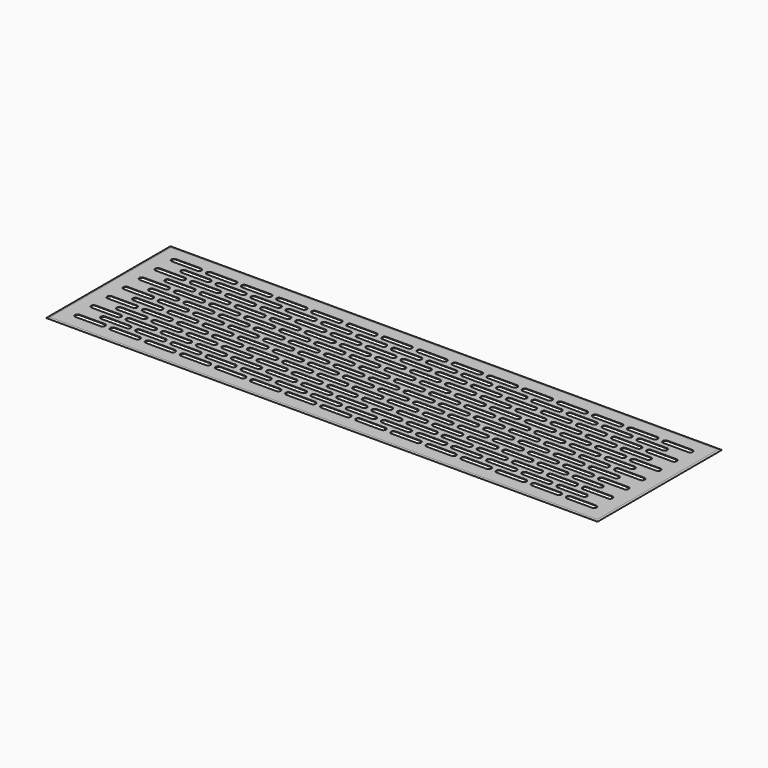
from build123d import *

# Parameters (mm, degrees)
F0_W        = 550
F0_H        = 155
F1_DEPTH    = 0.5
F3_DEPTH    = 0.5
F5_DEPTH    = 0.5
F6_T1_DEPTH = 165.8972473589
F6_T3_DEPTH = 560.8972473589


# Not quite as in the source:
# - a fillet or chamfer that OpenCascade refuses, or shapes differently, is made with other operations: its cross-section is extruded or revolved along the edge and cut away or added


with BuildPart() as f1:
    # F0 (on Top) → F1 (new body)
    with BuildSketch(Plane.XY):
        with Locations((45.4935486417, 1.9829720259)):
            Rectangle(F0_W, F0_H)
    extrude(amount=F1_DEPTH)

    # F2 (on face) → F3 (cut)
    with BuildSketch(Plane.XY.offset(0.5)):
        with BuildLine():
            Line((-187.0064513583, 44.4829720259), (-212.0064513583, 44.4829720259))
            ThreePointArc((-212.0064513583, 44.4829720259), (-213.7742183113, 43.7507389788), (-214.5064513583, 41.9829720259))
            ThreePointArc((-214.5064513583, 41.9829720259), (-213.7742183113, 40.2152050729), (-212.0064513583, 39.4829720259))
            Line((-212.0064513583, 39.4829720259), (-187.0064513583, 39.4829720259))
            ThreePointArc((-187.0064513583, 39.4829720259), (-185.2386844053, 40.2152050729), (-184.5064513583, 41.9829720259))
            ThreePointArc((-184.5064513583, 41.9829720259), (-185.2386844053, 43.7507389788), (-187.0064513583, 44.4829720259))
        make_face()
        with BuildLine():
            Line((-187.0064513583, 64.4829720259), (-212.0064513583, 64.4829720259))
            ThreePointArc((-212.0064513583, 64.4829720259), (-213.7742183113, 63.7507389788), (-214.5064513583, 61.9829720259))
            ThreePointArc((-214.5064513583, 61.9829720259), (-213.7742183113, 60.2152050729), (-212.0064513583, 59.4829720259))
            Line((-212.0064513583, 59.4829720259), (-187.0064513583, 59.4829720259))
            ThreePointArc((-187.0064513583, 59.4829720259), (-185.2386844053, 60.2152050729), (-184.5064513583, 61.9829720259))
            ThreePointArc((-184.5064513583, 61.9829720259), (-185.2386844053, 63.7507389788), (-187.0064513583, 64.4829720259))
        make_face()
        with BuildLine():
            Line((-152.0064513583, -55.5170279741), (-177.0064513583, -55.5170279741))
            ThreePointArc((-177.0064513583, -55.5170279741), (-178.7742183113, -56.2492610212), (-179.5064513583, -58.0170279741))
            ThreePointArc((-179.5064513583, -58.0170279741), (-178.7742183113, -59.7847949271), (-177.0064513583, -60.5170279741))
            Line((-177.0064513583, -60.5170279741), (-152.0064513583, -60.5170279741))
            ThreePointArc((-152.0064513583, -60.5170279741), (-150.2386844053, -59.7847949271), (-149.5064513583, -58.0170279741))
            ThreePointArc((-149.5064513583, -58.0170279741), (-150.2386844053, -56.2492610212), (-152.0064513583, -55.5170279741))
        make_face()
        with BuildLine():
            Line((-152.0064513583, -15.5170279741), (-177.0064513583, -15.5170279741))
            ThreePointArc((-177.0064513583, -15.5170279741), (-178.7742183113, -16.2492610212), (-179.5064513583, -18.0170279741))
            ThreePointArc((-179.5064513583, -18.0170279741), (-178.7742183113, -19.7847949271), (-177.0064513583, -20.5170279741))
            Line((-177.0064513583, -20.5170279741), (-152.0064513583, -20.5170279741))
            ThreePointArc((-152.0064513583, -20.5170279741), (-150.2386844053, -19.7847949271), (-149.5064513583, -18.0170279741))
            ThreePointArc((-149.5064513583, -18.0170279741), (-150.2386844053, -16.2492610212), (-152.0064513583, -15.5170279741))
        make_face()
        with BuildLine():
            Line((-152.0064513583, 24.4829720259), (-177.0064513583, 24.4829720259))
            ThreePointArc((-177.0064513583, 24.4829720259), (-178.7742183113, 23.7507389788), (-179.5064513583, 21.9829720259))
            ThreePointArc((-179.5064513583, 21.9829720259), (-178.7742183113, 20.2152050729), (-177.0064513583, 19.4829720259))
            Line((-177.0064513583, 19.4829720259), (-152.0064513583, 19.4829720259))
            ThreePointArc((-152.0064513583, 19.4829720259), (-150.2386844053, 20.2152050729), (-149.5064513583, 21.9829720259))
            ThreePointArc((-149.5064513583, 21.9829720259), (-150.2386844053, 23.7507389788), (-152.0064513583, 24.4829720259))
        make_face()
        with BuildLine():
            Line((-152.0064513583, 4.4829720259), (-177.0064513583, 4.4829720259))
            ThreePointArc((-177.0064513583, 4.4829720259), (-178.7742183113, 3.7507389788), (-179.5064513583, 1.9829720259))
            ThreePointArc((-179.5064513583, 1.9829720259), (-178.7742183113, 0.2152050729), (-177.0064513583, -0.5170279741))
            Line((-177.0064513583, -0.5170279741), (-152.0064513583, -0.5170279741))
            ThreePointArc((-152.0064513583, -0.5170279741), (-150.2386844053, 0.2152050729), (-149.5064513583, 1.9829720259))
            ThreePointArc((-149.5064513583, 1.9829720259), (-150.2386844053, 3.7507389788), (-152.0064513583, 4.4829720259))
        make_face()
        with BuildLine():
            Line((-152.0064513583, 44.4829720259), (-177.0064513583, 44.4829720259))
            ThreePointArc((-177.0064513583, 44.4829720259), (-178.7742183113, 43.7507389788), (-179.5064513583, 41.9829720259))
            ThreePointArc((-179.5064513583, 41.9829720259), (-178.7742183113, 40.2152050729), (-177.0064513583, 39.4829720259))
            Line((-177.0064513583, 39.4829720259), (-152.0064513583, 39.4829720259))
            ThreePointArc((-152.0064513583, 39.4829720259), (-150.2386844053, 40.2152050729), (-149.5064513583, 41.9829720259))
            ThreePointArc((-149.5064513583, 41.9829720259), (-150.2386844053, 43.7507389788), (-152.0064513583, 44.4829720259))
        make_face()
        with BuildLine():
            Line((-187.0064513583, 24.4829720259), (-212.0064513583, 24.4829720259))
            ThreePointArc((-212.0064513583, 24.4829720259), (-213.7742183113, 23.7507389788), (-214.5064513583, 21.9829720259))
            ThreePointArc((-214.5064513583, 21.9829720259), (-213.7742183113, 20.2152050729), (-212.0064513583, 19.4829720259))
            Line((-212.0064513583, 19.4829720259), (-187.0064513583, 19.4829720259))
            ThreePointArc((-187.0064513583, 19.4829720259), (-185.2386844053, 20.2152050729), (-184.5064513583, 21.9829720259))
            ThreePointArc((-184.5064513583, 21.9829720259), (-185.2386844053, 23.7507389788), (-187.0064513583, 24.4829720259))
        make_face()
        with BuildLine():
            Line((-187.0064513583, 4.4829720259), (-212.0064513583, 4.4829720259))
            ThreePointArc((-212.0064513583, 4.4829720259), (-213.7742183113, 3.7507389788), (-214.5064513583, 1.9829720259))
            ThreePointArc((-214.5064513583, 1.9829720259), (-213.7742183113, 0.2152050729), (-212.0064513583, -0.5170279741))
            Line((-212.0064513583, -0.5170279741), (-187.0064513583, -0.5170279741))
            ThreePointArc((-187.0064513583, -0.5170279741), (-185.2386844053, 0.2152050729), (-184.5064513583, 1.9829720259))
            ThreePointArc((-184.5064513583, 1.9829720259), (-185.2386844053, 3.7507389788), (-187.0064513583, 4.4829720259))
        make_face()
        with BuildLine():
            Line((-187.0064513583, -15.5170279741), (-212.0064513583, -15.5170279741))
            ThreePointArc((-212.0064513583, -15.5170279741), (-213.7742183113, -16.2492610212), (-214.5064513583, -18.0170279741))
            ThreePointArc((-214.5064513583, -18.0170279741), (-213.7742183113, -19.7847949271), (-212.0064513583, -20.5170279741))
            Line((-212.0064513583, -20.5170279741), (-187.0064513583, -20.5170279741))
            ThreePointArc((-187.0064513583, -20.5170279741), (-185.2386844053, -19.7847949271), (-184.5064513583, -18.0170279741))
            ThreePointArc((-184.5064513583, -18.0170279741), (-185.2386844053, -16.2492610212), (-187.0064513583, -15.5170279741))
        make_face()
        with BuildLine():
            Line((-187.0064513583, -35.5170279741), (-212.0064513583, -35.5170279741))
            ThreePointArc((-212.0064513583, -35.5170279741), (-213.7742183113, -36.2492610212), (-214.5064513583, -38.0170279741))
            ThreePointArc((-214.5064513583, -38.0170279741), (-213.7742183113, -39.7847949271), (-212.0064513583, -40.5170279741))
            Line((-212.0064513583, -40.5170279741), (-187.0064513583, -40.5170279741))
            ThreePointArc((-187.0064513583, -40.5170279741), (-185.2386844053, -39.7847949271), (-184.5064513583, -38.0170279741))
            ThreePointArc((-184.5064513583, -38.0170279741), (-185.2386844053, -36.2492610212), (-187.0064513583, -35.5170279741))
        make_face()
        with BuildLine():
            Line((-187.0064513583, -55.5170279741), (-212.0064513583, -55.5170279741))
            ThreePointArc((-212.0064513583, -55.5170279741), (-213.7742183113, -56.2492610212), (-214.5064513583, -58.0170279741))
            ThreePointArc((-214.5064513583, -58.0170279741), (-213.7742183113, -59.7847949271), (-212.0064513583, -60.5170279741))
            Line((-212.0064513583, -60.5170279741), (-187.0064513583, -60.5170279741))
            ThreePointArc((-187.0064513583, -60.5170279741), (-185.2386844053, -59.7847949271), (-184.5064513583, -58.0170279741))
            ThreePointArc((-184.5064513583, -58.0170279741), (-185.2386844053, -56.2492610212), (-187.0064513583, -55.5170279741))
        make_face()
        with BuildLine():
            Line((-117.0064513583, -55.5170279741), (-142.0064513583, -55.5170279741))
            ThreePointArc((-142.0064513583, -55.5170279741), (-143.7742183113, -56.2492610212), (-144.5064513583, -58.0170279741))
            ThreePointArc((-144.5064513583, -58.0170279741), (-143.7742183113, -59.7847949271), (-142.0064513583, -60.5170279741))
            Line((-142.0064513583, -60.5170279741), (-117.0064513583, -60.5170279741))
            ThreePointArc((-117.0064513583, -60.5170279741), (-115.2386844053, -59.7847949271), (-114.5064513583, -58.0170279741))
            ThreePointArc((-114.5064513583, -58.0170279741), (-115.2386844053, -56.2492610212), (-117.0064513583, -55.5170279741))
        make_face()
        with BuildLine():
            Line((-152.0064513583, 64.4829720259), (-177.0064513583, 64.4829720259))
            ThreePointArc((-177.0064513583, 64.4829720259), (-178.7742183113, 63.7507389788), (-179.5064513583, 61.9829720259))
            ThreePointArc((-179.5064513583, 61.9829720259), (-178.7742183113, 60.2152050729), (-177.0064513583, 59.4829720259))
            Line((-177.0064513583, 59.4829720259), (-152.0064513583, 59.4829720259))
            ThreePointArc((-152.0064513583, 59.4829720259), (-150.2386844053, 60.2152050729), (-149.5064513583, 61.9829720259))
            ThreePointArc((-149.5064513583, 61.9829720259), (-150.2386844053, 63.7507389788), (-152.0064513583, 64.4829720259))
        make_face()
        with BuildLine():
            Line((-117.0064513583, -35.5170279741), (-142.0064513583, -35.5170279741))
            ThreePointArc((-142.0064513583, -35.5170279741), (-143.7742183113, -36.2492610212), (-144.5064513583, -38.0170279741))
            ThreePointArc((-144.5064513583, -38.0170279741), (-143.7742183113, -39.7847949271), (-142.0064513583, -40.5170279741))
            Line((-142.0064513583, -40.5170279741), (-117.0064513583, -40.5170279741))
            ThreePointArc((-117.0064513583, -40.5170279741), (-115.2386844053, -39.7847949271), (-114.5064513583, -38.0170279741))
            ThreePointArc((-114.5064513583, -38.0170279741), (-115.2386844053, -36.2492610212), (-117.0064513583, -35.5170279741))
        make_face()
        with BuildLine():
            Line((-152.0064513583, -35.5170279741), (-177.0064513583, -35.5170279741))
            ThreePointArc((-177.0064513583, -35.5170279741), (-178.7742183113, -36.2492610212), (-179.5064513583, -38.0170279741))
            ThreePointArc((-179.5064513583, -38.0170279741), (-178.7742183113, -39.7847949271), (-177.0064513583, -40.5170279741))
            Line((-177.0064513583, -40.5170279741), (-152.0064513583, -40.5170279741))
            ThreePointArc((-152.0064513583, -40.5170279741), (-150.2386844053, -39.7847949271), (-149.5064513583, -38.0170279741))
            ThreePointArc((-149.5064513583, -38.0170279741), (-150.2386844053, -36.2492610212), (-152.0064513583, -35.5170279741))
        make_face()
        with BuildLine():
            Line((267.9935486417, -35.5170279741), (242.9935486417, -35.5170279741))
            ThreePointArc((242.9935486417, -35.5170279741), (241.2257816887, -36.2492610212), (240.4935486417, -38.0170279741))
            ThreePointArc((240.4935486417, -38.0170279741), (241.2257816887, -39.7847949271), (242.9935486417, -40.5170279741))
            Line((242.9935486417, -40.5170279741), (267.9935486417, -40.5170279741))
            ThreePointArc((267.9935486417, -40.5170279741), (269.7613155947, -39.7847949271), (270.4935486417, -38.0170279741))
            ThreePointArc((270.4935486417, -38.0170279741), (269.7613155947, -36.2492610212), (267.9935486417, -35.5170279741))
        make_face()
        with BuildLine():
            Line((-47.0064513583, -55.5170279741), (-72.0064513583, -55.5170279741))
            ThreePointArc((-72.0064513583, -55.5170279741), (-73.7742183113, -56.2492610212), (-74.5064513583, -58.0170279741))
            ThreePointArc((-74.5064513583, -58.0170279741), (-73.7742183113, -59.7847949271), (-72.0064513583, -60.5170279741))
            Line((-72.0064513583, -60.5170279741), (-47.0064513583, -60.5170279741))
            ThreePointArc((-47.0064513583, -60.5170279741), (-45.2386844053, -59.7847949271), (-44.5064513583, -58.0170279741))
            ThreePointArc((-44.5064513583, -58.0170279741), (-45.2386844053, -56.2492610212), (-47.0064513583, -55.5170279741))
        make_face()
        with BuildLine():
            Line((22.9935486417, -15.5170279741), (-2.0064513583, -15.5170279741))
            ThreePointArc((-2.0064513583, -15.5170279741), (-3.7742183113, -16.2492610212), (-4.5064513583, -18.0170279741))
            ThreePointArc((-4.5064513583, -18.0170279741), (-3.7742183113, -19.7847949271), (-2.0064513583, -20.5170279741))
            Line((-2.0064513583, -20.5170279741), (22.9935486417, -20.5170279741))
            ThreePointArc((22.9935486417, -20.5170279741), (24.7613155947, -19.7847949271), (25.4935486417, -18.0170279741))
            ThreePointArc((25.4935486417, -18.0170279741), (24.7613155947, -16.2492610212), (22.9935486417, -15.5170279741))
        make_face()
        with BuildLine():
            Line((92.9935486417, 24.4829720259), (67.9935486417, 24.4829720259))
            ThreePointArc((67.9935486417, 24.4829720259), (66.2257816887, 23.7507389788), (65.4935486417, 21.9829720259))
            ThreePointArc((65.4935486417, 21.9829720259), (66.2257816887, 20.2152050729), (67.9935486417, 19.4829720259))
            Line((67.9935486417, 19.4829720259), (92.9935486417, 19.4829720259))
            ThreePointArc((92.9935486417, 19.4829720259), (94.7613155947, 20.2152050729), (95.4935486417, 21.9829720259))
            ThreePointArc((95.4935486417, 21.9829720259), (94.7613155947, 23.7507389788), (92.9935486417, 24.4829720259))
        make_face()
        with BuildLine():
            Line((162.9935486417, 64.4829720259), (137.9935486417, 64.4829720259))
            ThreePointArc((137.9935486417, 64.4829720259), (136.2257816887, 63.7507389788), (135.4935486417, 61.9829720259))
            ThreePointArc((135.4935486417, 61.9829720259), (136.2257816887, 60.2152050729), (137.9935486417, 59.4829720259))
            Line((137.9935486417, 59.4829720259), (162.9935486417, 59.4829720259))
            ThreePointArc((162.9935486417, 59.4829720259), (164.7613155947, 60.2152050729), (165.4935486417, 61.9829720259))
            ThreePointArc((165.4935486417, 61.9829720259), (164.7613155947, 63.7507389788), (162.9935486417, 64.4829720259))
        make_face()
        with BuildLine():
            Line((267.9935486417, -55.5170279741), (242.9935486417, -55.5170279741))
            ThreePointArc((242.9935486417, -55.5170279741), (241.2257816887, -56.2492610212), (240.4935486417, -58.0170279741))
            ThreePointArc((240.4935486417, -58.0170279741), (241.2257816887, -59.7847949271), (242.9935486417, -60.5170279741))
            Line((242.9935486417, -60.5170279741), (267.9935486417, -60.5170279741))
            ThreePointArc((267.9935486417, -60.5170279741), (269.7613155947, -59.7847949271), (270.4935486417, -58.0170279741))
            ThreePointArc((270.4935486417, -58.0170279741), (269.7613155947, -56.2492610212), (267.9935486417, -55.5170279741))
        make_face()
        with BuildLine():
            Line((-82.0064513583, 64.4829720259), (-107.0064513583, 64.4829720259))
            ThreePointArc((-107.0064513583, 64.4829720259), (-108.7742183113, 63.7507389788), (-109.5064513583, 61.9829720259))
            ThreePointArc((-109.5064513583, 61.9829720259), (-108.7742183113, 60.2152050729), (-107.0064513583, 59.4829720259))
            Line((-107.0064513583, 59.4829720259), (-82.0064513583, 59.4829720259))
            ThreePointArc((-82.0064513583, 59.4829720259), (-80.2386844053, 60.2152050729), (-79.5064513583, 61.9829720259))
            ThreePointArc((-79.5064513583, 61.9829720259), (-80.2386844053, 63.7507389788), (-82.0064513583, 64.4829720259))
        make_face()
        with BuildLine():
            Line((22.9935486417, -35.5170279741), (-2.0064513583, -35.5170279741))
            ThreePointArc((-2.0064513583, -35.5170279741), (-3.7742183113, -36.2492610212), (-4.5064513583, -38.0170279741))
            ThreePointArc((-4.5064513583, -38.0170279741), (-3.7742183113, -39.7847949271), (-2.0064513583, -40.5170279741))
            Line((-2.0064513583, -40.5170279741), (22.9935486417, -40.5170279741))
            ThreePointArc((22.9935486417, -40.5170279741), (24.7613155947, -39.7847949271), (25.4935486417, -38.0170279741))
            ThreePointArc((25.4935486417, -38.0170279741), (24.7613155947, -36.2492610212), (22.9935486417, -35.5170279741))
        make_face()
        with BuildLine():
            Line((92.9935486417, 4.4829720259), (67.9935486417, 4.4829720259))
            ThreePointArc((67.9935486417, 4.4829720259), (66.2257816887, 3.7507389788), (65.4935486417, 1.9829720259))
            ThreePointArc((65.4935486417, 1.9829720259), (66.2257816887, 0.2152050729), (67.9935486417, -0.5170279741))
            Line((67.9935486417, -0.5170279741), (92.9935486417, -0.5170279741))
            ThreePointArc((92.9935486417, -0.5170279741), (94.7613155947, 0.2152050729), (95.4935486417, 1.9829720259))
            ThreePointArc((95.4935486417, 1.9829720259), (94.7613155947, 3.7507389788), (92.9935486417, 4.4829720259))
        make_face()
        with BuildLine():
            Line((162.9935486417, 44.4829720259), (137.9935486417, 44.4829720259))
            ThreePointArc((137.9935486417, 44.4829720259), (136.2257816887, 43.7507389788), (135.4935486417, 41.9829720259))
            ThreePointArc((135.4935486417, 41.9829720259), (136.2257816887, 40.2152050729), (137.9935486417, 39.4829720259))
            Line((137.9935486417, 39.4829720259), (162.9935486417, 39.4829720259))
            ThreePointArc((162.9935486417, 39.4829720259), (164.7613155947, 40.2152050729), (165.4935486417, 41.9829720259))
            ThreePointArc((165.4935486417, 41.9829720259), (164.7613155947, 43.7507389788), (162.9935486417, 44.4829720259))
        make_face()
        with BuildLine():
            Line((232.9935486417, 64.4829720259), (207.9935486417, 64.4829720259))
            ThreePointArc((207.9935486417, 64.4829720259), (206.2257816887, 63.7507389788), (205.4935486417, 61.9829720259))
            ThreePointArc((205.4935486417, 61.9829720259), (206.2257816887, 60.2152050729), (207.9935486417, 59.4829720259))
            Line((207.9935486417, 59.4829720259), (232.9935486417, 59.4829720259))
            ThreePointArc((232.9935486417, 59.4829720259), (234.7613155947, 60.2152050729), (235.4935486417, 61.9829720259))
            ThreePointArc((235.4935486417, 61.9829720259), (234.7613155947, 63.7507389788), (232.9935486417, 64.4829720259))
        make_face()
        with BuildLine():
            Line((-82.0064513583, 44.4829720259), (-107.0064513583, 44.4829720259))
            ThreePointArc((-107.0064513583, 44.4829720259), (-108.7742183113, 43.7507389788), (-109.5064513583, 41.9829720259))
            ThreePointArc((-109.5064513583, 41.9829720259), (-108.7742183113, 40.2152050729), (-107.0064513583, 39.4829720259))
            Line((-107.0064513583, 39.4829720259), (-82.0064513583, 39.4829720259))
            ThreePointArc((-82.0064513583, 39.4829720259), (-80.2386844053, 40.2152050729), (-79.5064513583, 41.9829720259))
            ThreePointArc((-79.5064513583, 41.9829720259), (-80.2386844053, 43.7507389788), (-82.0064513583, 44.4829720259))
        make_face()
        with BuildLine():
            Line((22.9935486417, -55.5170279741), (-2.0064513583, -55.5170279741))
            ThreePointArc((-2.0064513583, -55.5170279741), (-3.7742183113, -56.2492610212), (-4.5064513583, -58.0170279741))
            ThreePointArc((-4.5064513583, -58.0170279741), (-3.7742183113, -59.7847949271), (-2.0064513583, -60.5170279741))
            Line((-2.0064513583, -60.5170279741), (22.9935486417, -60.5170279741))
            ThreePointArc((22.9935486417, -60.5170279741), (24.7613155947, -59.7847949271), (25.4935486417, -58.0170279741))
            ThreePointArc((25.4935486417, -58.0170279741), (24.7613155947, -56.2492610212), (22.9935486417, -55.5170279741))
        make_face()
        with BuildLine():
            Line((92.9935486417, -15.5170279741), (67.9935486417, -15.5170279741))
            ThreePointArc((67.9935486417, -15.5170279741), (66.2257816887, -16.2492610212), (65.4935486417, -18.0170279741))
            ThreePointArc((65.4935486417, -18.0170279741), (66.2257816887, -19.7847949271), (67.9935486417, -20.5170279741))
            Line((67.9935486417, -20.5170279741), (92.9935486417, -20.5170279741))
            ThreePointArc((92.9935486417, -20.5170279741), (94.7613155947, -19.7847949271), (95.4935486417, -18.0170279741))
            ThreePointArc((95.4935486417, -18.0170279741), (94.7613155947, -16.2492610212), (92.9935486417, -15.5170279741))
        make_face()
        with BuildLine():
            Line((162.9935486417, 24.4829720259), (137.9935486417, 24.4829720259))
            ThreePointArc((137.9935486417, 24.4829720259), (136.2257816887, 23.7507389788), (135.4935486417, 21.9829720259))
            ThreePointArc((135.4935486417, 21.9829720259), (136.2257816887, 20.2152050729), (137.9935486417, 19.4829720259))
            Line((137.9935486417, 19.4829720259), (162.9935486417, 19.4829720259))
            ThreePointArc((162.9935486417, 19.4829720259), (164.7613155947, 20.2152050729), (165.4935486417, 21.9829720259))
            ThreePointArc((165.4935486417, 21.9829720259), (164.7613155947, 23.7507389788), (162.9935486417, 24.4829720259))
        make_face()
        with BuildLine():
            Line((232.9935486417, 44.4829720259), (207.9935486417, 44.4829720259))
            ThreePointArc((207.9935486417, 44.4829720259), (206.2257816887, 43.7507389788), (205.4935486417, 41.9829720259))
            ThreePointArc((205.4935486417, 41.9829720259), (206.2257816887, 40.2152050729), (207.9935486417, 39.4829720259))
            Line((207.9935486417, 39.4829720259), (232.9935486417, 39.4829720259))
            ThreePointArc((232.9935486417, 39.4829720259), (234.7613155947, 40.2152050729), (235.4935486417, 41.9829720259))
            ThreePointArc((235.4935486417, 41.9829720259), (234.7613155947, 43.7507389788), (232.9935486417, 44.4829720259))
        make_face()
        with BuildLine():
            Line((-82.0064513583, 24.4829720259), (-107.0064513583, 24.4829720259))
            ThreePointArc((-107.0064513583, 24.4829720259), (-108.7742183113, 23.7507389788), (-109.5064513583, 21.9829720259))
            ThreePointArc((-109.5064513583, 21.9829720259), (-108.7742183113, 20.2152050729), (-107.0064513583, 19.4829720259))
            Line((-107.0064513583, 19.4829720259), (-82.0064513583, 19.4829720259))
            ThreePointArc((-82.0064513583, 19.4829720259), (-80.2386844053, 20.2152050729), (-79.5064513583, 21.9829720259))
            ThreePointArc((-79.5064513583, 21.9829720259), (-80.2386844053, 23.7507389788), (-82.0064513583, 24.4829720259))
        make_face()
        with BuildLine():
            Line((-12.0064513583, 64.4829720259), (-37.0064513583, 64.4829720259))
            ThreePointArc((-37.0064513583, 64.4829720259), (-38.7742183113, 63.7507389788), (-39.5064513583, 61.9829720259))
            ThreePointArc((-39.5064513583, 61.9829720259), (-38.7742183113, 60.2152050729), (-37.0064513583, 59.4829720259))
            Line((-37.0064513583, 59.4829720259), (-12.0064513583, 59.4829720259))
            ThreePointArc((-12.0064513583, 59.4829720259), (-10.2386844053, 60.2152050729), (-9.5064513583, 61.9829720259))
            ThreePointArc((-9.5064513583, 61.9829720259), (-10.2386844053, 63.7507389788), (-12.0064513583, 64.4829720259))
        make_face()
        with BuildLine():
            Line((92.9935486417, -35.5170279741), (67.9935486417, -35.5170279741))
            ThreePointArc((67.9935486417, -35.5170279741), (66.2257816887, -36.2492610212), (65.4935486417, -38.0170279741))
            ThreePointArc((65.4935486417, -38.0170279741), (66.2257816887, -39.7847949271), (67.9935486417, -40.5170279741))
            Line((67.9935486417, -40.5170279741), (92.9935486417, -40.5170279741))
            ThreePointArc((92.9935486417, -40.5170279741), (94.7613155947, -39.7847949271), (95.4935486417, -38.0170279741))
            ThreePointArc((95.4935486417, -38.0170279741), (94.7613155947, -36.2492610212), (92.9935486417, -35.5170279741))
        make_face()
        with BuildLine():
            Line((162.9935486417, 4.4829720259), (137.9935486417, 4.4829720259))
            ThreePointArc((137.9935486417, 4.4829720259), (136.2257816887, 3.7507389788), (135.4935486417, 1.9829720259))
            ThreePointArc((135.4935486417, 1.9829720259), (136.2257816887, 0.2152050729), (137.9935486417, -0.5170279741))
            Line((137.9935486417, -0.5170279741), (162.9935486417, -0.5170279741))
            ThreePointArc((162.9935486417, -0.5170279741), (164.7613155947, 0.2152050729), (165.4935486417, 1.9829720259))
            ThreePointArc((165.4935486417, 1.9829720259), (164.7613155947, 3.7507389788), (162.9935486417, 4.4829720259))
        make_face()
        with BuildLine():
            Line((232.9935486417, 24.4829720259), (207.9935486417, 24.4829720259))
            ThreePointArc((207.9935486417, 24.4829720259), (206.2257816887, 23.7507389788), (205.4935486417, 21.9829720259))
            ThreePointArc((205.4935486417, 21.9829720259), (206.2257816887, 20.2152050729), (207.9935486417, 19.4829720259))
            Line((207.9935486417, 19.4829720259), (232.9935486417, 19.4829720259))
            ThreePointArc((232.9935486417, 19.4829720259), (234.7613155947, 20.2152050729), (235.4935486417, 21.9829720259))
            ThreePointArc((235.4935486417, 21.9829720259), (234.7613155947, 23.7507389788), (232.9935486417, 24.4829720259))
        make_face()
        with BuildLine():
            Line((302.9935486417, 64.4829720259), (277.9935486417, 64.4829720259))
            ThreePointArc((277.9935486417, 64.4829720259), (276.2257816887, 63.7507389788), (275.4935486417, 61.9829720259))
            ThreePointArc((275.4935486417, 61.9829720259), (276.2257816887, 60.2152050729), (277.9935486417, 59.4829720259))
            Line((277.9935486417, 59.4829720259), (302.9935486417, 59.4829720259))
            ThreePointArc((302.9935486417, 59.4829720259), (304.7613155947, 60.2152050729), (305.4935486417, 61.9829720259))
            ThreePointArc((305.4935486417, 61.9829720259), (304.7613155947, 63.7507389788), (302.9935486417, 64.4829720259))
        make_face()
        with BuildLine():
            Line((-82.0064513583, 4.4829720259), (-107.0064513583, 4.4829720259))
            ThreePointArc((-107.0064513583, 4.4829720259), (-108.7742183113, 3.7507389788), (-109.5064513583, 1.9829720259))
            ThreePointArc((-109.5064513583, 1.9829720259), (-108.7742183113, 0.2152050729), (-107.0064513583, -0.5170279741))
            Line((-107.0064513583, -0.5170279741), (-82.0064513583, -0.5170279741))
            ThreePointArc((-82.0064513583, -0.5170279741), (-80.2386844053, 0.2152050729), (-79.5064513583, 1.9829720259))
            ThreePointArc((-79.5064513583, 1.9829720259), (-80.2386844053, 3.7507389788), (-82.0064513583, 4.4829720259))
        make_face()
        with BuildLine():
            Line((-12.0064513583, 44.4829720259), (-37.0064513583, 44.4829720259))
            ThreePointArc((-37.0064513583, 44.4829720259), (-38.7742183113, 43.7507389788), (-39.5064513583, 41.9829720259))
            ThreePointArc((-39.5064513583, 41.9829720259), (-38.7742183113, 40.2152050729), (-37.0064513583, 39.4829720259))
            Line((-37.0064513583, 39.4829720259), (-12.0064513583, 39.4829720259))
            ThreePointArc((-12.0064513583, 39.4829720259), (-10.2386844053, 40.2152050729), (-9.5064513583, 41.9829720259))
            ThreePointArc((-9.5064513583, 41.9829720259), (-10.2386844053, 43.7507389788), (-12.0064513583, 44.4829720259))
        make_face()
        with BuildLine():
            Line((92.9935486417, -55.5170279741), (67.9935486417, -55.5170279741))
            ThreePointArc((67.9935486417, -55.5170279741), (66.2257816887, -56.2492610212), (65.4935486417, -58.0170279741))
            ThreePointArc((65.4935486417, -58.0170279741), (66.2257816887, -59.7847949271), (67.9935486417, -60.5170279741))
            Line((67.9935486417, -60.5170279741), (92.9935486417, -60.5170279741))
            ThreePointArc((92.9935486417, -60.5170279741), (94.7613155947, -59.7847949271), (95.4935486417, -58.0170279741))
            ThreePointArc((95.4935486417, -58.0170279741), (94.7613155947, -56.2492610212), (92.9935486417, -55.5170279741))
        make_face()
        with BuildLine():
            Line((162.9935486417, -15.5170279741), (137.9935486417, -15.5170279741))
            ThreePointArc((137.9935486417, -15.5170279741), (136.2257816887, -16.2492610212), (135.4935486417, -18.0170279741))
            ThreePointArc((135.4935486417, -18.0170279741), (136.2257816887, -19.7847949271), (137.9935486417, -20.5170279741))
            Line((137.9935486417, -20.5170279741), (162.9935486417, -20.5170279741))
            ThreePointArc((162.9935486417, -20.5170279741), (164.7613155947, -19.7847949271), (165.4935486417, -18.0170279741))
            ThreePointArc((165.4935486417, -18.0170279741), (164.7613155947, -16.2492610212), (162.9935486417, -15.5170279741))
        make_face()
        with BuildLine():
            Line((-82.0064513583, -15.5170279741), (-107.0064513583, -15.5170279741))
            ThreePointArc((-107.0064513583, -15.5170279741), (-108.7742183113, -16.2492610212), (-109.5064513583, -18.0170279741))
            ThreePointArc((-109.5064513583, -18.0170279741), (-108.7742183113, -19.7847949271), (-107.0064513583, -20.5170279741))
            Line((-107.0064513583, -20.5170279741), (-82.0064513583, -20.5170279741))
            ThreePointArc((-82.0064513583, -20.5170279741), (-80.2386844053, -19.7847949271), (-79.5064513583, -18.0170279741))
            ThreePointArc((-79.5064513583, -18.0170279741), (-80.2386844053, -16.2492610212), (-82.0064513583, -15.5170279741))
        make_face()
        with BuildLine():
            Line((-12.0064513583, 24.4829720259), (-37.0064513583, 24.4829720259))
            ThreePointArc((-37.0064513583, 24.4829720259), (-38.7742183113, 23.7507389788), (-39.5064513583, 21.9829720259))
            ThreePointArc((-39.5064513583, 21.9829720259), (-38.7742183113, 20.2152050729), (-37.0064513583, 19.4829720259))
            Line((-37.0064513583, 19.4829720259), (-12.0064513583, 19.4829720259))
            ThreePointArc((-12.0064513583, 19.4829720259), (-10.2386844053, 20.2152050729), (-9.5064513583, 21.9829720259))
            ThreePointArc((-9.5064513583, 21.9829720259), (-10.2386844053, 23.7507389788), (-12.0064513583, 24.4829720259))
        make_face()
        with BuildLine():
            Line((57.9935486417, 64.4829720259), (32.9935486417, 64.4829720259))
            ThreePointArc((32.9935486417, 64.4829720259), (31.2257816887, 63.7507389788), (30.4935486417, 61.9829720259))
            ThreePointArc((30.4935486417, 61.9829720259), (31.2257816887, 60.2152050729), (32.9935486417, 59.4829720259))
            Line((32.9935486417, 59.4829720259), (57.9935486417, 59.4829720259))
            ThreePointArc((57.9935486417, 59.4829720259), (59.7613155947, 60.2152050729), (60.4935486417, 61.9829720259))
            ThreePointArc((60.4935486417, 61.9829720259), (59.7613155947, 63.7507389788), (57.9935486417, 64.4829720259))
        make_face()
        with BuildLine():
            Line((162.9935486417, -35.5170279741), (137.9935486417, -35.5170279741))
            ThreePointArc((137.9935486417, -35.5170279741), (136.2257816887, -36.2492610212), (135.4935486417, -38.0170279741))
            ThreePointArc((135.4935486417, -38.0170279741), (136.2257816887, -39.7847949271), (137.9935486417, -40.5170279741))
            Line((137.9935486417, -40.5170279741), (162.9935486417, -40.5170279741))
            ThreePointArc((162.9935486417, -40.5170279741), (164.7613155947, -39.7847949271), (165.4935486417, -38.0170279741))
            ThreePointArc((165.4935486417, -38.0170279741), (164.7613155947, -36.2492610212), (162.9935486417, -35.5170279741))
        make_face()
        with BuildLine():
            Line((232.9935486417, 4.4829720259), (207.9935486417, 4.4829720259))
            ThreePointArc((207.9935486417, 4.4829720259), (206.2257816887, 3.7507389788), (205.4935486417, 1.9829720259))
            ThreePointArc((205.4935486417, 1.9829720259), (206.2257816887, 0.2152050729), (207.9935486417, -0.5170279741))
            Line((207.9935486417, -0.5170279741), (232.9935486417, -0.5170279741))
            ThreePointArc((232.9935486417, -0.5170279741), (234.7613155947, 0.2152050729), (235.4935486417, 1.9829720259))
            ThreePointArc((235.4935486417, 1.9829720259), (234.7613155947, 3.7507389788), (232.9935486417, 4.4829720259))
        make_face()
        with BuildLine():
            Line((302.9935486417, 44.4829720259), (277.9935486417, 44.4829720259))
            ThreePointArc((277.9935486417, 44.4829720259), (276.2257816887, 43.7507389788), (275.4935486417, 41.9829720259))
            ThreePointArc((275.4935486417, 41.9829720259), (276.2257816887, 40.2152050729), (277.9935486417, 39.4829720259))
            Line((277.9935486417, 39.4829720259), (302.9935486417, 39.4829720259))
            ThreePointArc((302.9935486417, 39.4829720259), (304.7613155947, 40.2152050729), (305.4935486417, 41.9829720259))
            ThreePointArc((305.4935486417, 41.9829720259), (304.7613155947, 43.7507389788), (302.9935486417, 44.4829720259))
        make_face()
        with BuildLine():
            Line((232.9935486417, -15.5170279741), (207.9935486417, -15.5170279741))
            ThreePointArc((207.9935486417, -15.5170279741), (206.2257816887, -16.2492610212), (205.4935486417, -18.0170279741))
            ThreePointArc((205.4935486417, -18.0170279741), (206.2257816887, -19.7847949271), (207.9935486417, -20.5170279741))
            Line((207.9935486417, -20.5170279741), (232.9935486417, -20.5170279741))
            ThreePointArc((232.9935486417, -20.5170279741), (234.7613155947, -19.7847949271), (235.4935486417, -18.0170279741))
            ThreePointArc((235.4935486417, -18.0170279741), (234.7613155947, -16.2492610212), (232.9935486417, -15.5170279741))
        make_face()
        with BuildLine():
            Line((302.9935486417, 24.4829720259), (277.9935486417, 24.4829720259))
            ThreePointArc((277.9935486417, 24.4829720259), (276.2257816887, 23.7507389788), (275.4935486417, 21.9829720259))
            ThreePointArc((275.4935486417, 21.9829720259), (276.2257816887, 20.2152050729), (277.9935486417, 19.4829720259))
            Line((277.9935486417, 19.4829720259), (302.9935486417, 19.4829720259))
            ThreePointArc((302.9935486417, 19.4829720259), (304.7613155947, 20.2152050729), (305.4935486417, 21.9829720259))
            ThreePointArc((305.4935486417, 21.9829720259), (304.7613155947, 23.7507389788), (302.9935486417, 24.4829720259))
        make_face()
        with BuildLine():
            Line((-82.0064513583, -35.5170279741), (-107.0064513583, -35.5170279741))
            ThreePointArc((-107.0064513583, -35.5170279741), (-108.7742183113, -36.2492610212), (-109.5064513583, -38.0170279741))
            ThreePointArc((-109.5064513583, -38.0170279741), (-108.7742183113, -39.7847949271), (-107.0064513583, -40.5170279741))
            Line((-107.0064513583, -40.5170279741), (-82.0064513583, -40.5170279741))
            ThreePointArc((-82.0064513583, -40.5170279741), (-80.2386844053, -39.7847949271), (-79.5064513583, -38.0170279741))
            ThreePointArc((-79.5064513583, -38.0170279741), (-80.2386844053, -36.2492610212), (-82.0064513583, -35.5170279741))
        make_face()
        with BuildLine():
            Line((-12.0064513583, 4.4829720259), (-37.0064513583, 4.4829720259))
            ThreePointArc((-37.0064513583, 4.4829720259), (-38.7742183113, 3.7507389788), (-39.5064513583, 1.9829720259))
            ThreePointArc((-39.5064513583, 1.9829720259), (-38.7742183113, 0.2152050729), (-37.0064513583, -0.5170279741))
            Line((-37.0064513583, -0.5170279741), (-12.0064513583, -0.5170279741))
            ThreePointArc((-12.0064513583, -0.5170279741), (-10.2386844053, 0.2152050729), (-9.5064513583, 1.9829720259))
            ThreePointArc((-9.5064513583, 1.9829720259), (-10.2386844053, 3.7507389788), (-12.0064513583, 4.4829720259))
        make_face()
        with BuildLine():
            Line((57.9935486417, 44.4829720259), (32.9935486417, 44.4829720259))
            ThreePointArc((32.9935486417, 44.4829720259), (31.2257816887, 43.7507389788), (30.4935486417, 41.9829720259))
            ThreePointArc((30.4935486417, 41.9829720259), (31.2257816887, 40.2152050729), (32.9935486417, 39.4829720259))
            Line((32.9935486417, 39.4829720259), (57.9935486417, 39.4829720259))
            ThreePointArc((57.9935486417, 39.4829720259), (59.7613155947, 40.2152050729), (60.4935486417, 41.9829720259))
            ThreePointArc((60.4935486417, 41.9829720259), (59.7613155947, 43.7507389788), (57.9935486417, 44.4829720259))
        make_face()
        with BuildLine():
            Line((162.9935486417, -55.5170279741), (137.9935486417, -55.5170279741))
            ThreePointArc((137.9935486417, -55.5170279741), (136.2257816887, -56.2492610212), (135.4935486417, -58.0170279741))
            ThreePointArc((135.4935486417, -58.0170279741), (136.2257816887, -59.7847949271), (137.9935486417, -60.5170279741))
            Line((137.9935486417, -60.5170279741), (162.9935486417, -60.5170279741))
            ThreePointArc((162.9935486417, -60.5170279741), (164.7613155947, -59.7847949271), (165.4935486417, -58.0170279741))
            ThreePointArc((165.4935486417, -58.0170279741), (164.7613155947, -56.2492610212), (162.9935486417, -55.5170279741))
        make_face()
        with BuildLine():
            Line((57.9935486417, 24.4829720259), (32.9935486417, 24.4829720259))
            ThreePointArc((32.9935486417, 24.4829720259), (31.2257816887, 23.7507389788), (30.4935486417, 21.9829720259))
            ThreePointArc((30.4935486417, 21.9829720259), (31.2257816887, 20.2152050729), (32.9935486417, 19.4829720259))
            Line((32.9935486417, 19.4829720259), (57.9935486417, 19.4829720259))
            ThreePointArc((57.9935486417, 19.4829720259), (59.7613155947, 20.2152050729), (60.4935486417, 21.9829720259))
            ThreePointArc((60.4935486417, 21.9829720259), (59.7613155947, 23.7507389788), (57.9935486417, 24.4829720259))
        make_face()
        with BuildLine():
            Line((127.9935486417, 64.4829720259), (102.9935486417, 64.4829720259))
            ThreePointArc((102.9935486417, 64.4829720259), (101.2257816887, 63.7507389788), (100.4935486417, 61.9829720259))
            ThreePointArc((100.4935486417, 61.9829720259), (101.2257816887, 60.2152050729), (102.9935486417, 59.4829720259))
            Line((102.9935486417, 59.4829720259), (127.9935486417, 59.4829720259))
            ThreePointArc((127.9935486417, 59.4829720259), (129.7613155947, 60.2152050729), (130.4935486417, 61.9829720259))
            ThreePointArc((130.4935486417, 61.9829720259), (129.7613155947, 63.7507389788), (127.9935486417, 64.4829720259))
        make_face()
        with BuildLine():
            Line((232.9935486417, -35.5170279741), (207.9935486417, -35.5170279741))
            ThreePointArc((207.9935486417, -35.5170279741), (206.2257816887, -36.2492610212), (205.4935486417, -38.0170279741))
            ThreePointArc((205.4935486417, -38.0170279741), (206.2257816887, -39.7847949271), (207.9935486417, -40.5170279741))
            Line((207.9935486417, -40.5170279741), (232.9935486417, -40.5170279741))
            ThreePointArc((232.9935486417, -40.5170279741), (234.7613155947, -39.7847949271), (235.4935486417, -38.0170279741))
            ThreePointArc((235.4935486417, -38.0170279741), (234.7613155947, -36.2492610212), (232.9935486417, -35.5170279741))
        make_face()
        with BuildLine():
            Line((302.9935486417, 4.4829720259), (277.9935486417, 4.4829720259))
            ThreePointArc((277.9935486417, 4.4829720259), (276.2257816887, 3.7507389788), (275.4935486417, 1.9829720259))
            ThreePointArc((275.4935486417, 1.9829720259), (276.2257816887, 0.2152050729), (277.9935486417, -0.5170279741))
            Line((277.9935486417, -0.5170279741), (302.9935486417, -0.5170279741))
            ThreePointArc((302.9935486417, -0.5170279741), (304.7613155947, 0.2152050729), (305.4935486417, 1.9829720259))
            ThreePointArc((305.4935486417, 1.9829720259), (304.7613155947, 3.7507389788), (302.9935486417, 4.4829720259))
        make_face()
        with BuildLine():
            Line((-82.0064513583, -55.5170279741), (-107.0064513583, -55.5170279741))
            ThreePointArc((-107.0064513583, -55.5170279741), (-108.7742183113, -56.2492610212), (-109.5064513583, -58.0170279741))
            ThreePointArc((-109.5064513583, -58.0170279741), (-108.7742183113, -59.7847949271), (-107.0064513583, -60.5170279741))
            Line((-107.0064513583, -60.5170279741), (-82.0064513583, -60.5170279741))
            ThreePointArc((-82.0064513583, -60.5170279741), (-80.2386844053, -59.7847949271), (-79.5064513583, -58.0170279741))
            ThreePointArc((-79.5064513583, -58.0170279741), (-80.2386844053, -56.2492610212), (-82.0064513583, -55.5170279741))
        make_face()
        with BuildLine():
            Line((-12.0064513583, -15.5170279741), (-37.0064513583, -15.5170279741))
            ThreePointArc((-37.0064513583, -15.5170279741), (-38.7742183113, -16.2492610212), (-39.5064513583, -18.0170279741))
            ThreePointArc((-39.5064513583, -18.0170279741), (-38.7742183113, -19.7847949271), (-37.0064513583, -20.5170279741))
            Line((-37.0064513583, -20.5170279741), (-12.0064513583, -20.5170279741))
            ThreePointArc((-12.0064513583, -20.5170279741), (-10.2386844053, -19.7847949271), (-9.5064513583, -18.0170279741))
            ThreePointArc((-9.5064513583, -18.0170279741), (-10.2386844053, -16.2492610212), (-12.0064513583, -15.5170279741))
        make_face()
        with BuildLine():
            Line((57.9935486417, 4.4829720259), (32.9935486417, 4.4829720259))
            ThreePointArc((32.9935486417, 4.4829720259), (31.2257816887, 3.7507389788), (30.4935486417, 1.9829720259))
            ThreePointArc((30.4935486417, 1.9829720259), (31.2257816887, 0.2152050729), (32.9935486417, -0.5170279741))
            Line((32.9935486417, -0.5170279741), (57.9935486417, -0.5170279741))
            ThreePointArc((57.9935486417, -0.5170279741), (59.7613155947, 0.2152050729), (60.4935486417, 1.9829720259))
            ThreePointArc((60.4935486417, 1.9829720259), (59.7613155947, 3.7507389788), (57.9935486417, 4.4829720259))
        make_face()
        with BuildLine():
            Line((127.9935486417, 44.4829720259), (102.9935486417, 44.4829720259))
            ThreePointArc((102.9935486417, 44.4829720259), (101.2257816887, 43.7507389788), (100.4935486417, 41.9829720259))
            ThreePointArc((100.4935486417, 41.9829720259), (101.2257816887, 40.2152050729), (102.9935486417, 39.4829720259))
            Line((102.9935486417, 39.4829720259), (127.9935486417, 39.4829720259))
            ThreePointArc((127.9935486417, 39.4829720259), (129.7613155947, 40.2152050729), (130.4935486417, 41.9829720259))
            ThreePointArc((130.4935486417, 41.9829720259), (129.7613155947, 43.7507389788), (127.9935486417, 44.4829720259))
        make_face()
        with BuildLine():
            Line((232.9935486417, -55.5170279741), (207.9935486417, -55.5170279741))
            ThreePointArc((207.9935486417, -55.5170279741), (206.2257816887, -56.2492610212), (205.4935486417, -58.0170279741))
            ThreePointArc((205.4935486417, -58.0170279741), (206.2257816887, -59.7847949271), (207.9935486417, -60.5170279741))
            Line((207.9935486417, -60.5170279741), (232.9935486417, -60.5170279741))
            ThreePointArc((232.9935486417, -60.5170279741), (234.7613155947, -59.7847949271), (235.4935486417, -58.0170279741))
            ThreePointArc((235.4935486417, -58.0170279741), (234.7613155947, -56.2492610212), (232.9935486417, -55.5170279741))
        make_face()
        with BuildLine():
            Line((302.9935486417, -15.5170279741), (277.9935486417, -15.5170279741))
            ThreePointArc((277.9935486417, -15.5170279741), (276.2257816887, -16.2492610212), (275.4935486417, -18.0170279741))
            ThreePointArc((275.4935486417, -18.0170279741), (276.2257816887, -19.7847949271), (277.9935486417, -20.5170279741))
            Line((277.9935486417, -20.5170279741), (302.9935486417, -20.5170279741))
            ThreePointArc((302.9935486417, -20.5170279741), (304.7613155947, -19.7847949271), (305.4935486417, -18.0170279741))
            ThreePointArc((305.4935486417, -18.0170279741), (304.7613155947, -16.2492610212), (302.9935486417, -15.5170279741))
        make_face()
        with BuildLine():
            Line((-117.0064513583, 64.4829720259), (-142.0064513583, 64.4829720259))
            ThreePointArc((-142.0064513583, 64.4829720259), (-143.7742183113, 63.7507389788), (-144.5064513583, 61.9829720259))
            ThreePointArc((-144.5064513583, 61.9829720259), (-143.7742183113, 60.2152050729), (-142.0064513583, 59.4829720259))
            Line((-142.0064513583, 59.4829720259), (-117.0064513583, 59.4829720259))
            ThreePointArc((-117.0064513583, 59.4829720259), (-115.2386844053, 60.2152050729), (-114.5064513583, 61.9829720259))
            ThreePointArc((-114.5064513583, 61.9829720259), (-115.2386844053, 63.7507389788), (-117.0064513583, 64.4829720259))
        make_face()
        with BuildLine():
            Line((-12.0064513583, -35.5170279741), (-37.0064513583, -35.5170279741))
            ThreePointArc((-37.0064513583, -35.5170279741), (-38.7742183113, -36.2492610212), (-39.5064513583, -38.0170279741))
            ThreePointArc((-39.5064513583, -38.0170279741), (-38.7742183113, -39.7847949271), (-37.0064513583, -40.5170279741))
            Line((-37.0064513583, -40.5170279741), (-12.0064513583, -40.5170279741))
            ThreePointArc((-12.0064513583, -40.5170279741), (-10.2386844053, -39.7847949271), (-9.5064513583, -38.0170279741))
            ThreePointArc((-9.5064513583, -38.0170279741), (-10.2386844053, -36.2492610212), (-12.0064513583, -35.5170279741))
        make_face()
        with BuildLine():
            Line((57.9935486417, -15.5170279741), (32.9935486417, -15.5170279741))
            ThreePointArc((32.9935486417, -15.5170279741), (31.2257816887, -16.2492610212), (30.4935486417, -18.0170279741))
            ThreePointArc((30.4935486417, -18.0170279741), (31.2257816887, -19.7847949271), (32.9935486417, -20.5170279741))
            Line((32.9935486417, -20.5170279741), (57.9935486417, -20.5170279741))
            ThreePointArc((57.9935486417, -20.5170279741), (59.7613155947, -19.7847949271), (60.4935486417, -18.0170279741))
            ThreePointArc((60.4935486417, -18.0170279741), (59.7613155947, -16.2492610212), (57.9935486417, -15.5170279741))
        make_face()
        with BuildLine():
            Line((127.9935486417, 24.4829720259), (102.9935486417, 24.4829720259))
            ThreePointArc((102.9935486417, 24.4829720259), (101.2257816887, 23.7507389788), (100.4935486417, 21.9829720259))
            ThreePointArc((100.4935486417, 21.9829720259), (101.2257816887, 20.2152050729), (102.9935486417, 19.4829720259))
            Line((102.9935486417, 19.4829720259), (127.9935486417, 19.4829720259))
            ThreePointArc((127.9935486417, 19.4829720259), (129.7613155947, 20.2152050729), (130.4935486417, 21.9829720259))
            ThreePointArc((130.4935486417, 21.9829720259), (129.7613155947, 23.7507389788), (127.9935486417, 24.4829720259))
        make_face()
        with BuildLine():
            Line((197.9935486417, 64.4829720259), (172.9935486417, 64.4829720259))
            ThreePointArc((172.9935486417, 64.4829720259), (171.2257816887, 63.7507389788), (170.4935486417, 61.9829720259))
            ThreePointArc((170.4935486417, 61.9829720259), (171.2257816887, 60.2152050729), (172.9935486417, 59.4829720259))
            Line((172.9935486417, 59.4829720259), (197.9935486417, 59.4829720259))
            ThreePointArc((197.9935486417, 59.4829720259), (199.7613155947, 60.2152050729), (200.4935486417, 61.9829720259))
            ThreePointArc((200.4935486417, 61.9829720259), (199.7613155947, 63.7507389788), (197.9935486417, 64.4829720259))
        make_face()
        with BuildLine():
            Line((302.9935486417, -35.5170279741), (277.9935486417, -35.5170279741))
            ThreePointArc((277.9935486417, -35.5170279741), (276.2257816887, -36.2492610212), (275.4935486417, -38.0170279741))
            ThreePointArc((275.4935486417, -38.0170279741), (276.2257816887, -39.7847949271), (277.9935486417, -40.5170279741))
            Line((277.9935486417, -40.5170279741), (302.9935486417, -40.5170279741))
            ThreePointArc((302.9935486417, -40.5170279741), (304.7613155947, -39.7847949271), (305.4935486417, -38.0170279741))
            ThreePointArc((305.4935486417, -38.0170279741), (304.7613155947, -36.2492610212), (302.9935486417, -35.5170279741))
        make_face()
        with BuildLine():
            Line((-117.0064513583, 44.4829720259), (-142.0064513583, 44.4829720259))
            ThreePointArc((-142.0064513583, 44.4829720259), (-143.7742183113, 43.7507389788), (-144.5064513583, 41.9829720259))
            ThreePointArc((-144.5064513583, 41.9829720259), (-143.7742183113, 40.2152050729), (-142.0064513583, 39.4829720259))
            Line((-142.0064513583, 39.4829720259), (-117.0064513583, 39.4829720259))
            ThreePointArc((-117.0064513583, 39.4829720259), (-115.2386844053, 40.2152050729), (-114.5064513583, 41.9829720259))
            ThreePointArc((-114.5064513583, 41.9829720259), (-115.2386844053, 43.7507389788), (-117.0064513583, 44.4829720259))
        make_face()
        with BuildLine():
            Line((-12.0064513583, -55.5170279741), (-37.0064513583, -55.5170279741))
            ThreePointArc((-37.0064513583, -55.5170279741), (-38.7742183113, -56.2492610212), (-39.5064513583, -58.0170279741))
            ThreePointArc((-39.5064513583, -58.0170279741), (-38.7742183113, -59.7847949271), (-37.0064513583, -60.5170279741))
            Line((-37.0064513583, -60.5170279741), (-12.0064513583, -60.5170279741))
            ThreePointArc((-12.0064513583, -60.5170279741), (-10.2386844053, -59.7847949271), (-9.5064513583, -58.0170279741))
            ThreePointArc((-9.5064513583, -58.0170279741), (-10.2386844053, -56.2492610212), (-12.0064513583, -55.5170279741))
        make_face()
        with BuildLine():
            Line((57.9935486417, -35.5170279741), (32.9935486417, -35.5170279741))
            ThreePointArc((32.9935486417, -35.5170279741), (31.2257816887, -36.2492610212), (30.4935486417, -38.0170279741))
            ThreePointArc((30.4935486417, -38.0170279741), (31.2257816887, -39.7847949271), (32.9935486417, -40.5170279741))
            Line((32.9935486417, -40.5170279741), (57.9935486417, -40.5170279741))
            ThreePointArc((57.9935486417, -40.5170279741), (59.7613155947, -39.7847949271), (60.4935486417, -38.0170279741))
            ThreePointArc((60.4935486417, -38.0170279741), (59.7613155947, -36.2492610212), (57.9935486417, -35.5170279741))
        make_face()
        with BuildLine():
            Line((127.9935486417, 4.4829720259), (102.9935486417, 4.4829720259))
            ThreePointArc((102.9935486417, 4.4829720259), (101.2257816887, 3.7507389788), (100.4935486417, 1.9829720259))
            ThreePointArc((100.4935486417, 1.9829720259), (101.2257816887, 0.2152050729), (102.9935486417, -0.5170279741))
            Line((102.9935486417, -0.5170279741), (127.9935486417, -0.5170279741))
            ThreePointArc((127.9935486417, -0.5170279741), (129.7613155947, 0.2152050729), (130.4935486417, 1.9829720259))
            ThreePointArc((130.4935486417, 1.9829720259), (129.7613155947, 3.7507389788), (127.9935486417, 4.4829720259))
        make_face()
        with BuildLine():
            Line((197.9935486417, 44.4829720259), (172.9935486417, 44.4829720259))
            ThreePointArc((172.9935486417, 44.4829720259), (171.2257816887, 43.7507389788), (170.4935486417, 41.9829720259))
            ThreePointArc((170.4935486417, 41.9829720259), (171.2257816887, 40.2152050729), (172.9935486417, 39.4829720259))
            Line((172.9935486417, 39.4829720259), (197.9935486417, 39.4829720259))
            ThreePointArc((197.9935486417, 39.4829720259), (199.7613155947, 40.2152050729), (200.4935486417, 41.9829720259))
            ThreePointArc((200.4935486417, 41.9829720259), (199.7613155947, 43.7507389788), (197.9935486417, 44.4829720259))
        make_face()
        with BuildLine():
            Line((302.9935486417, -55.5170279741), (277.9935486417, -55.5170279741))
            ThreePointArc((277.9935486417, -55.5170279741), (276.2257816887, -56.2492610212), (275.4935486417, -58.0170279741))
            ThreePointArc((275.4935486417, -58.0170279741), (276.2257816887, -59.7847949271), (277.9935486417, -60.5170279741))
            Line((277.9935486417, -60.5170279741), (302.9935486417, -60.5170279741))
            ThreePointArc((302.9935486417, -60.5170279741), (304.7613155947, -59.7847949271), (305.4935486417, -58.0170279741))
            ThreePointArc((305.4935486417, -58.0170279741), (304.7613155947, -56.2492610212), (302.9935486417, -55.5170279741))
        make_face()
        with BuildLine():
            Line((-117.0064513583, 24.4829720259), (-142.0064513583, 24.4829720259))
            ThreePointArc((-142.0064513583, 24.4829720259), (-143.7742183113, 23.7507389788), (-144.5064513583, 21.9829720259))
            ThreePointArc((-144.5064513583, 21.9829720259), (-143.7742183113, 20.2152050729), (-142.0064513583, 19.4829720259))
            Line((-142.0064513583, 19.4829720259), (-117.0064513583, 19.4829720259))
            ThreePointArc((-117.0064513583, 19.4829720259), (-115.2386844053, 20.2152050729), (-114.5064513583, 21.9829720259))
            ThreePointArc((-114.5064513583, 21.9829720259), (-115.2386844053, 23.7507389788), (-117.0064513583, 24.4829720259))
        make_face()
        with BuildLine():
            Line((-47.0064513583, 64.4829720259), (-72.0064513583, 64.4829720259))
            ThreePointArc((-72.0064513583, 64.4829720259), (-73.7742183113, 63.7507389788), (-74.5064513583, 61.9829720259))
            ThreePointArc((-74.5064513583, 61.9829720259), (-73.7742183113, 60.2152050729), (-72.0064513583, 59.4829720259))
            Line((-72.0064513583, 59.4829720259), (-47.0064513583, 59.4829720259))
            ThreePointArc((-47.0064513583, 59.4829720259), (-45.2386844053, 60.2152050729), (-44.5064513583, 61.9829720259))
            ThreePointArc((-44.5064513583, 61.9829720259), (-45.2386844053, 63.7507389788), (-47.0064513583, 64.4829720259))
        make_face()
        with BuildLine():
            Line((57.9935486417, -55.5170279741), (32.9935486417, -55.5170279741))
            ThreePointArc((32.9935486417, -55.5170279741), (31.2257816887, -56.2492610212), (30.4935486417, -58.0170279741))
            ThreePointArc((30.4935486417, -58.0170279741), (31.2257816887, -59.7847949271), (32.9935486417, -60.5170279741))
            Line((32.9935486417, -60.5170279741), (57.9935486417, -60.5170279741))
            ThreePointArc((57.9935486417, -60.5170279741), (59.7613155947, -59.7847949271), (60.4935486417, -58.0170279741))
            ThreePointArc((60.4935486417, -58.0170279741), (59.7613155947, -56.2492610212), (57.9935486417, -55.5170279741))
        make_face()
        with BuildLine():
            Line((127.9935486417, -15.5170279741), (102.9935486417, -15.5170279741))
            ThreePointArc((102.9935486417, -15.5170279741), (101.2257816887, -16.2492610212), (100.4935486417, -18.0170279741))
            ThreePointArc((100.4935486417, -18.0170279741), (101.2257816887, -19.7847949271), (102.9935486417, -20.5170279741))
            Line((102.9935486417, -20.5170279741), (127.9935486417, -20.5170279741))
            ThreePointArc((127.9935486417, -20.5170279741), (129.7613155947, -19.7847949271), (130.4935486417, -18.0170279741))
            ThreePointArc((130.4935486417, -18.0170279741), (129.7613155947, -16.2492610212), (127.9935486417, -15.5170279741))
        make_face()
        with BuildLine():
            Line((197.9935486417, 24.4829720259), (172.9935486417, 24.4829720259))
            ThreePointArc((172.9935486417, 24.4829720259), (171.2257816887, 23.7507389788), (170.4935486417, 21.9829720259))
            ThreePointArc((170.4935486417, 21.9829720259), (171.2257816887, 20.2152050729), (172.9935486417, 19.4829720259))
            Line((172.9935486417, 19.4829720259), (197.9935486417, 19.4829720259))
            ThreePointArc((197.9935486417, 19.4829720259), (199.7613155947, 20.2152050729), (200.4935486417, 21.9829720259))
            ThreePointArc((200.4935486417, 21.9829720259), (199.7613155947, 23.7507389788), (197.9935486417, 24.4829720259))
        make_face()
        with BuildLine():
            Line((267.9935486417, 64.4829720259), (242.9935486417, 64.4829720259))
            ThreePointArc((242.9935486417, 64.4829720259), (241.2257816887, 63.7507389788), (240.4935486417, 61.9829720259))
            ThreePointArc((240.4935486417, 61.9829720259), (241.2257816887, 60.2152050729), (242.9935486417, 59.4829720259))
            Line((242.9935486417, 59.4829720259), (267.9935486417, 59.4829720259))
            ThreePointArc((267.9935486417, 59.4829720259), (269.7613155947, 60.2152050729), (270.4935486417, 61.9829720259))
            ThreePointArc((270.4935486417, 61.9829720259), (269.7613155947, 63.7507389788), (267.9935486417, 64.4829720259))
        make_face()
        with BuildLine():
            Line((-117.0064513583, 4.4829720259), (-142.0064513583, 4.4829720259))
            ThreePointArc((-142.0064513583, 4.4829720259), (-143.7742183113, 3.7507389788), (-144.5064513583, 1.9829720259))
            ThreePointArc((-144.5064513583, 1.9829720259), (-143.7742183113, 0.2152050729), (-142.0064513583, -0.5170279741))
            Line((-142.0064513583, -0.5170279741), (-117.0064513583, -0.5170279741))
            ThreePointArc((-117.0064513583, -0.5170279741), (-115.2386844053, 0.2152050729), (-114.5064513583, 1.9829720259))
            ThreePointArc((-114.5064513583, 1.9829720259), (-115.2386844053, 3.7507389788), (-117.0064513583, 4.4829720259))
        make_face()
        with BuildLine():
            Line((-47.0064513583, 44.4829720259), (-72.0064513583, 44.4829720259))
            ThreePointArc((-72.0064513583, 44.4829720259), (-73.7742183113, 43.7507389788), (-74.5064513583, 41.9829720259))
            ThreePointArc((-74.5064513583, 41.9829720259), (-73.7742183113, 40.2152050729), (-72.0064513583, 39.4829720259))
            Line((-72.0064513583, 39.4829720259), (-47.0064513583, 39.4829720259))
            ThreePointArc((-47.0064513583, 39.4829720259), (-45.2386844053, 40.2152050729), (-44.5064513583, 41.9829720259))
            ThreePointArc((-44.5064513583, 41.9829720259), (-45.2386844053, 43.7507389788), (-47.0064513583, 44.4829720259))
        make_face()
        with BuildLine():
            Line((22.9935486417, 64.4829720259), (-2.0064513583, 64.4829720259))
            ThreePointArc((-2.0064513583, 64.4829720259), (-3.7742183113, 63.7507389788), (-4.5064513583, 61.9829720259))
            ThreePointArc((-4.5064513583, 61.9829720259), (-3.7742183113, 60.2152050729), (-2.0064513583, 59.4829720259))
            Line((-2.0064513583, 59.4829720259), (22.9935486417, 59.4829720259))
            ThreePointArc((22.9935486417, 59.4829720259), (24.7613155947, 60.2152050729), (25.4935486417, 61.9829720259))
            ThreePointArc((25.4935486417, 61.9829720259), (24.7613155947, 63.7507389788), (22.9935486417, 64.4829720259))
        make_face()
        with BuildLine():
            Line((197.9935486417, 4.4829720259), (172.9935486417, 4.4829720259))
            ThreePointArc((172.9935486417, 4.4829720259), (171.2257816887, 3.7507389788), (170.4935486417, 1.9829720259))
            ThreePointArc((170.4935486417, 1.9829720259), (171.2257816887, 0.2152050729), (172.9935486417, -0.5170279741))
            Line((172.9935486417, -0.5170279741), (197.9935486417, -0.5170279741))
            ThreePointArc((197.9935486417, -0.5170279741), (199.7613155947, 0.2152050729), (200.4935486417, 1.9829720259))
            ThreePointArc((200.4935486417, 1.9829720259), (199.7613155947, 3.7507389788), (197.9935486417, 4.4829720259))
        make_face()
        with BuildLine():
            Line((127.9935486417, -35.5170279741), (102.9935486417, -35.5170279741))
            ThreePointArc((102.9935486417, -35.5170279741), (101.2257816887, -36.2492610212), (100.4935486417, -38.0170279741))
            ThreePointArc((100.4935486417, -38.0170279741), (101.2257816887, -39.7847949271), (102.9935486417, -40.5170279741))
            Line((102.9935486417, -40.5170279741), (127.9935486417, -40.5170279741))
            ThreePointArc((127.9935486417, -40.5170279741), (129.7613155947, -39.7847949271), (130.4935486417, -38.0170279741))
            ThreePointArc((130.4935486417, -38.0170279741), (129.7613155947, -36.2492610212), (127.9935486417, -35.5170279741))
        make_face()
        with BuildLine():
            Line((267.9935486417, 44.4829720259), (242.9935486417, 44.4829720259))
            ThreePointArc((242.9935486417, 44.4829720259), (241.2257816887, 43.7507389788), (240.4935486417, 41.9829720259))
            ThreePointArc((240.4935486417, 41.9829720259), (241.2257816887, 40.2152050729), (242.9935486417, 39.4829720259))
            Line((242.9935486417, 39.4829720259), (267.9935486417, 39.4829720259))
            ThreePointArc((267.9935486417, 39.4829720259), (269.7613155947, 40.2152050729), (270.4935486417, 41.9829720259))
            ThreePointArc((270.4935486417, 41.9829720259), (269.7613155947, 43.7507389788), (267.9935486417, 44.4829720259))
        make_face()
        with BuildLine():
            Line((-117.0064513583, -15.5170279741), (-142.0064513583, -15.5170279741))
            ThreePointArc((-142.0064513583, -15.5170279741), (-143.7742183113, -16.2492610212), (-144.5064513583, -18.0170279741))
            ThreePointArc((-144.5064513583, -18.0170279741), (-143.7742183113, -19.7847949271), (-142.0064513583, -20.5170279741))
            Line((-142.0064513583, -20.5170279741), (-117.0064513583, -20.5170279741))
            ThreePointArc((-117.0064513583, -20.5170279741), (-115.2386844053, -19.7847949271), (-114.5064513583, -18.0170279741))
            ThreePointArc((-114.5064513583, -18.0170279741), (-115.2386844053, -16.2492610212), (-117.0064513583, -15.5170279741))
        make_face()
        with BuildLine():
            Line((-47.0064513583, 24.4829720259), (-72.0064513583, 24.4829720259))
            ThreePointArc((-72.0064513583, 24.4829720259), (-73.7742183113, 23.7507389788), (-74.5064513583, 21.9829720259))
            ThreePointArc((-74.5064513583, 21.9829720259), (-73.7742183113, 20.2152050729), (-72.0064513583, 19.4829720259))
            Line((-72.0064513583, 19.4829720259), (-47.0064513583, 19.4829720259))
            ThreePointArc((-47.0064513583, 19.4829720259), (-45.2386844053, 20.2152050729), (-44.5064513583, 21.9829720259))
            ThreePointArc((-44.5064513583, 21.9829720259), (-45.2386844053, 23.7507389788), (-47.0064513583, 24.4829720259))
        make_face()
        with BuildLine():
            Line((22.9935486417, 24.4829720259), (-2.0064513583, 24.4829720259))
            ThreePointArc((-2.0064513583, 24.4829720259), (-3.7742183113, 23.7507389788), (-4.5064513583, 21.9829720259))
            ThreePointArc((-4.5064513583, 21.9829720259), (-3.7742183113, 20.2152050729), (-2.0064513583, 19.4829720259))
            Line((-2.0064513583, 19.4829720259), (22.9935486417, 19.4829720259))
            ThreePointArc((22.9935486417, 19.4829720259), (24.7613155947, 20.2152050729), (25.4935486417, 21.9829720259))
            ThreePointArc((25.4935486417, 21.9829720259), (24.7613155947, 23.7507389788), (22.9935486417, 24.4829720259))
        make_face()
        with BuildLine():
            Line((92.9935486417, 64.4829720259), (67.9935486417, 64.4829720259))
            ThreePointArc((67.9935486417, 64.4829720259), (66.2257816887, 63.7507389788), (65.4935486417, 61.9829720259))
            ThreePointArc((65.4935486417, 61.9829720259), (66.2257816887, 60.2152050729), (67.9935486417, 59.4829720259))
            Line((67.9935486417, 59.4829720259), (92.9935486417, 59.4829720259))
            ThreePointArc((92.9935486417, 59.4829720259), (94.7613155947, 60.2152050729), (95.4935486417, 61.9829720259))
            ThreePointArc((95.4935486417, 61.9829720259), (94.7613155947, 63.7507389788), (92.9935486417, 64.4829720259))
        make_face()
        with BuildLine():
            Line((197.9935486417, -35.5170279741), (172.9935486417, -35.5170279741))
            ThreePointArc((172.9935486417, -35.5170279741), (171.2257816887, -36.2492610212), (170.4935486417, -38.0170279741))
            ThreePointArc((170.4935486417, -38.0170279741), (171.2257816887, -39.7847949271), (172.9935486417, -40.5170279741))
            Line((172.9935486417, -40.5170279741), (197.9935486417, -40.5170279741))
            ThreePointArc((197.9935486417, -40.5170279741), (199.7613155947, -39.7847949271), (200.4935486417, -38.0170279741))
            ThreePointArc((200.4935486417, -38.0170279741), (199.7613155947, -36.2492610212), (197.9935486417, -35.5170279741))
        make_face()
        with BuildLine():
            Line((267.9935486417, 4.4829720259), (242.9935486417, 4.4829720259))
            ThreePointArc((242.9935486417, 4.4829720259), (241.2257816887, 3.7507389788), (240.4935486417, 1.9829720259))
            ThreePointArc((240.4935486417, 1.9829720259), (241.2257816887, 0.2152050729), (242.9935486417, -0.5170279741))
            Line((242.9935486417, -0.5170279741), (267.9935486417, -0.5170279741))
            ThreePointArc((267.9935486417, -0.5170279741), (269.7613155947, 0.2152050729), (270.4935486417, 1.9829720259))
            ThreePointArc((270.4935486417, 1.9829720259), (269.7613155947, 3.7507389788), (267.9935486417, 4.4829720259))
        make_face()
        with BuildLine():
            Line((-47.0064513583, -15.5170279741), (-72.0064513583, -15.5170279741))
            ThreePointArc((-72.0064513583, -15.5170279741), (-73.7742183113, -16.2492610212), (-74.5064513583, -18.0170279741))
            ThreePointArc((-74.5064513583, -18.0170279741), (-73.7742183113, -19.7847949271), (-72.0064513583, -20.5170279741))
            Line((-72.0064513583, -20.5170279741), (-47.0064513583, -20.5170279741))
            ThreePointArc((-47.0064513583, -20.5170279741), (-45.2386844053, -19.7847949271), (-44.5064513583, -18.0170279741))
            ThreePointArc((-44.5064513583, -18.0170279741), (-45.2386844053, -16.2492610212), (-47.0064513583, -15.5170279741))
        make_face()
        with BuildLine():
            Line((22.9935486417, 4.4829720259), (-2.0064513583, 4.4829720259))
            ThreePointArc((-2.0064513583, 4.4829720259), (-3.7742183113, 3.7507389788), (-4.5064513583, 1.9829720259))
            ThreePointArc((-4.5064513583, 1.9829720259), (-3.7742183113, 0.2152050729), (-2.0064513583, -0.5170279741))
            Line((-2.0064513583, -0.5170279741), (22.9935486417, -0.5170279741))
            ThreePointArc((22.9935486417, -0.5170279741), (24.7613155947, 0.2152050729), (25.4935486417, 1.9829720259))
            ThreePointArc((25.4935486417, 1.9829720259), (24.7613155947, 3.7507389788), (22.9935486417, 4.4829720259))
        make_face()
        with BuildLine():
            Line((92.9935486417, 44.4829720259), (67.9935486417, 44.4829720259))
            ThreePointArc((67.9935486417, 44.4829720259), (66.2257816887, 43.7507389788), (65.4935486417, 41.9829720259))
            ThreePointArc((65.4935486417, 41.9829720259), (66.2257816887, 40.2152050729), (67.9935486417, 39.4829720259))
            Line((67.9935486417, 39.4829720259), (92.9935486417, 39.4829720259))
            ThreePointArc((92.9935486417, 39.4829720259), (94.7613155947, 40.2152050729), (95.4935486417, 41.9829720259))
            ThreePointArc((95.4935486417, 41.9829720259), (94.7613155947, 43.7507389788), (92.9935486417, 44.4829720259))
        make_face()
        with BuildLine():
            Line((197.9935486417, -55.5170279741), (172.9935486417, -55.5170279741))
            ThreePointArc((172.9935486417, -55.5170279741), (171.2257816887, -56.2492610212), (170.4935486417, -58.0170279741))
            ThreePointArc((170.4935486417, -58.0170279741), (171.2257816887, -59.7847949271), (172.9935486417, -60.5170279741))
            Line((172.9935486417, -60.5170279741), (197.9935486417, -60.5170279741))
            ThreePointArc((197.9935486417, -60.5170279741), (199.7613155947, -59.7847949271), (200.4935486417, -58.0170279741))
            ThreePointArc((200.4935486417, -58.0170279741), (199.7613155947, -56.2492610212), (197.9935486417, -55.5170279741))
        make_face()
        with BuildLine():
            Line((267.9935486417, -15.5170279741), (242.9935486417, -15.5170279741))
            ThreePointArc((242.9935486417, -15.5170279741), (241.2257816887, -16.2492610212), (240.4935486417, -18.0170279741))
            ThreePointArc((240.4935486417, -18.0170279741), (241.2257816887, -19.7847949271), (242.9935486417, -20.5170279741))
            Line((242.9935486417, -20.5170279741), (267.9935486417, -20.5170279741))
            ThreePointArc((267.9935486417, -20.5170279741), (269.7613155947, -19.7847949271), (270.4935486417, -18.0170279741))
            ThreePointArc((270.4935486417, -18.0170279741), (269.7613155947, -16.2492610212), (267.9935486417, -15.5170279741))
        make_face()
        with BuildLine():
            Line((-47.0064513583, -35.5170279741), (-72.0064513583, -35.5170279741))
            ThreePointArc((-72.0064513583, -35.5170279741), (-73.7742183113, -36.2492610212), (-74.5064513583, -38.0170279741))
            ThreePointArc((-74.5064513583, -38.0170279741), (-73.7742183113, -39.7847949271), (-72.0064513583, -40.5170279741))
            Line((-72.0064513583, -40.5170279741), (-47.0064513583, -40.5170279741))
            ThreePointArc((-47.0064513583, -40.5170279741), (-45.2386844053, -39.7847949271), (-44.5064513583, -38.0170279741))
            ThreePointArc((-44.5064513583, -38.0170279741), (-45.2386844053, -36.2492610212), (-47.0064513583, -35.5170279741))
        make_face()
        with BuildLine():
            Line((127.9935486417, -55.5170279741), (102.9935486417, -55.5170279741))
            ThreePointArc((102.9935486417, -55.5170279741), (101.2257816887, -56.2492610212), (100.4935486417, -58.0170279741))
            ThreePointArc((100.4935486417, -58.0170279741), (101.2257816887, -59.7847949271), (102.9935486417, -60.5170279741))
            Line((102.9935486417, -60.5170279741), (127.9935486417, -60.5170279741))
            ThreePointArc((127.9935486417, -60.5170279741), (129.7613155947, -59.7847949271), (130.4935486417, -58.0170279741))
            ThreePointArc((130.4935486417, -58.0170279741), (129.7613155947, -56.2492610212), (127.9935486417, -55.5170279741))
        make_face()
        with BuildLine():
            Line((197.9935486417, -15.5170279741), (172.9935486417, -15.5170279741))
            ThreePointArc((172.9935486417, -15.5170279741), (171.2257816887, -16.2492610212), (170.4935486417, -18.0170279741))
            ThreePointArc((170.4935486417, -18.0170279741), (171.2257816887, -19.7847949271), (172.9935486417, -20.5170279741))
            Line((172.9935486417, -20.5170279741), (197.9935486417, -20.5170279741))
            ThreePointArc((197.9935486417, -20.5170279741), (199.7613155947, -19.7847949271), (200.4935486417, -18.0170279741))
            ThreePointArc((200.4935486417, -18.0170279741), (199.7613155947, -16.2492610212), (197.9935486417, -15.5170279741))
        make_face()
        with BuildLine():
            Line((267.9935486417, 24.4829720259), (242.9935486417, 24.4829720259))
            ThreePointArc((242.9935486417, 24.4829720259), (241.2257816887, 23.7507389788), (240.4935486417, 21.9829720259))
            ThreePointArc((240.4935486417, 21.9829720259), (241.2257816887, 20.2152050729), (242.9935486417, 19.4829720259))
            Line((242.9935486417, 19.4829720259), (267.9935486417, 19.4829720259))
            ThreePointArc((267.9935486417, 19.4829720259), (269.7613155947, 20.2152050729), (270.4935486417, 21.9829720259))
            ThreePointArc((270.4935486417, 21.9829720259), (269.7613155947, 23.7507389788), (267.9935486417, 24.4829720259))
        make_face()
        with BuildLine():
            Line((-47.0064513583, 4.4829720259), (-72.0064513583, 4.4829720259))
            ThreePointArc((-72.0064513583, 4.4829720259), (-73.7742183113, 3.7507389788), (-74.5064513583, 1.9829720259))
            ThreePointArc((-74.5064513583, 1.9829720259), (-73.7742183113, 0.2152050729), (-72.0064513583, -0.5170279741))
            Line((-72.0064513583, -0.5170279741), (-47.0064513583, -0.5170279741))
            ThreePointArc((-47.0064513583, -0.5170279741), (-45.2386844053, 0.2152050729), (-44.5064513583, 1.9829720259))
            ThreePointArc((-44.5064513583, 1.9829720259), (-45.2386844053, 3.7507389788), (-47.0064513583, 4.4829720259))
        make_face()
        with BuildLine():
            Line((22.9935486417, 44.4829720259), (-2.0064513583, 44.4829720259))
            ThreePointArc((-2.0064513583, 44.4829720259), (-3.7742183113, 43.7507389788), (-4.5064513583, 41.9829720259))
            ThreePointArc((-4.5064513583, 41.9829720259), (-3.7742183113, 40.2152050729), (-2.0064513583, 39.4829720259))
            Line((-2.0064513583, 39.4829720259), (22.9935486417, 39.4829720259))
            ThreePointArc((22.9935486417, 39.4829720259), (24.7613155947, 40.2152050729), (25.4935486417, 41.9829720259))
            ThreePointArc((25.4935486417, 41.9829720259), (24.7613155947, 43.7507389788), (22.9935486417, 44.4829720259))
        make_face()
    extrude(amount=-F3_DEPTH, mode=Mode.SUBTRACT)

    # F4 (on face) → F5 (cut)
    with BuildSketch(Plane.XY.offset(0.5)):
        with BuildLine():
            ThreePointArc((47.9935486417, 51.9829720259), (48.7257816887, 50.2152050729), (50.4935486417, 49.4829720259))
            Line((50.4935486417, 49.4829720259), (75.4935486417, 49.4829720259))
            ThreePointArc((75.4935486417, 49.4829720259), (77.2613155947, 50.2152050729), (77.9935486417, 51.9829720259))
            ThreePointArc((77.9935486417, 51.9829720259), (77.2613155947, 53.7507389788), (75.4935486417, 54.4829720259))
            Line((75.4935486417, 54.4829720259), (50.4935486417, 54.4829720259))
            ThreePointArc((50.4935486417, 54.4829720259), (48.7257816887, 53.7507389788), (47.9935486417, 51.9829720259))
        make_face()
        with BuildLine():
            ThreePointArc((-57.0064513583, 51.9829720259), (-56.2742183113, 50.2152050729), (-54.5064513583, 49.4829720259))
            Line((-54.5064513583, 49.4829720259), (-29.5064513583, 49.4829720259))
            ThreePointArc((-29.5064513583, 49.4829720259), (-27.7386844053, 50.2152050729), (-27.0064513583, 51.9829720259))
            ThreePointArc((-27.0064513583, 51.9829720259), (-27.7386844053, 53.7507389788), (-29.5064513583, 54.4829720259))
            Line((-29.5064513583, 54.4829720259), (-54.5064513583, 54.4829720259))
            ThreePointArc((-54.5064513583, 54.4829720259), (-56.2742183113, 53.7507389788), (-57.0064513583, 51.9829720259))
        make_face()
        with BuildLine():
            ThreePointArc((222.9935486417, 51.9829720259), (223.7257816887, 50.2152050729), (225.4935486417, 49.4829720259))
            Line((225.4935486417, 49.4829720259), (250.4935486417, 49.4829720259))
            ThreePointArc((250.4935486417, 49.4829720259), (252.2613155947, 50.2152050729), (252.9935486417, 51.9829720259))
            ThreePointArc((252.9935486417, 51.9829720259), (252.2613155947, 53.7507389788), (250.4935486417, 54.4829720259))
            Line((250.4935486417, 54.4829720259), (225.4935486417, 54.4829720259))
            ThreePointArc((225.4935486417, 54.4829720259), (223.7257816887, 53.7507389788), (222.9935486417, 51.9829720259))
        make_face()
        with BuildLine():
            ThreePointArc((-127.0064513583, 51.9829720259), (-126.2742183113, 50.2152050729), (-124.5064513583, 49.4829720259))
            Line((-124.5064513583, 49.4829720259), (-99.5064513583, 49.4829720259))
            ThreePointArc((-99.5064513583, 49.4829720259), (-97.7386844053, 50.2152050729), (-97.0064513583, 51.9829720259))
            ThreePointArc((-97.0064513583, 51.9829720259), (-97.7386844053, 53.7507389788), (-99.5064513583, 54.4829720259))
            Line((-99.5064513583, 54.4829720259), (-124.5064513583, 54.4829720259))
            ThreePointArc((-124.5064513583, 54.4829720259), (-126.2742183113, 53.7507389788), (-127.0064513583, 51.9829720259))
        make_face()
        with BuildLine():
            ThreePointArc((152.9935486417, 51.9829720259), (153.7257816887, 50.2152050729), (155.4935486417, 49.4829720259))
            Line((155.4935486417, 49.4829720259), (180.4935486417, 49.4829720259))
            ThreePointArc((180.4935486417, 49.4829720259), (182.2613155947, 50.2152050729), (182.9935486417, 51.9829720259))
            ThreePointArc((182.9935486417, 51.9829720259), (182.2613155947, 53.7507389788), (180.4935486417, 54.4829720259))
            Line((180.4935486417, 54.4829720259), (155.4935486417, 54.4829720259))
            ThreePointArc((155.4935486417, 54.4829720259), (153.7257816887, 53.7507389788), (152.9935486417, 51.9829720259))
        make_face()
        with BuildLine():
            ThreePointArc((-22.0064513583, 51.9829720259), (-21.2742183113, 50.2152050729), (-19.5064513583, 49.4829720259))
            Line((-19.5064513583, 49.4829720259), (5.4935486417, 49.4829720259))
            ThreePointArc((5.4935486417, 49.4829720259), (7.2613155947, 50.2152050729), (7.9935486417, 51.9829720259))
            ThreePointArc((7.9935486417, 51.9829720259), (7.2613155947, 53.7507389788), (5.4935486417, 54.4829720259))
            Line((5.4935486417, 54.4829720259), (-19.5064513583, 54.4829720259))
            ThreePointArc((-19.5064513583, 54.4829720259), (-21.2742183113, 53.7507389788), (-22.0064513583, 51.9829720259))
        make_face()
        with BuildLine():
            ThreePointArc((257.9935486417, 51.9829720259), (258.7257816887, 50.2152050729), (260.4935486417, 49.4829720259))
            Line((260.4935486417, 49.4829720259), (285.4935486417, 49.4829720259))
            ThreePointArc((285.4935486417, 49.4829720259), (287.2613155947, 50.2152050729), (287.9935486417, 51.9829720259))
            ThreePointArc((287.9935486417, 51.9829720259), (287.2613155947, 53.7507389788), (285.4935486417, 54.4829720259))
            Line((285.4935486417, 54.4829720259), (260.4935486417, 54.4829720259))
            ThreePointArc((260.4935486417, 54.4829720259), (258.7257816887, 53.7507389788), (257.9935486417, 51.9829720259))
        make_face()
        with BuildLine():
            ThreePointArc((82.9935486417, 51.9829720259), (83.7257816887, 50.2152050729), (85.4935486417, 49.4829720259))
            Line((85.4935486417, 49.4829720259), (110.4935486417, 49.4829720259))
            ThreePointArc((110.4935486417, 49.4829720259), (112.2613155947, 50.2152050729), (112.9935486417, 51.9829720259))
            ThreePointArc((112.9935486417, 51.9829720259), (112.2613155947, 53.7507389788), (110.4935486417, 54.4829720259))
            Line((110.4935486417, 54.4829720259), (85.4935486417, 54.4829720259))
            ThreePointArc((85.4935486417, 54.4829720259), (83.7257816887, 53.7507389788), (82.9935486417, 51.9829720259))
        make_face()
        with BuildLine():
            ThreePointArc((187.9935486417, 51.9829720259), (188.7257816887, 50.2152050729), (190.4935486417, 49.4829720259))
            Line((190.4935486417, 49.4829720259), (215.4935486417, 49.4829720259))
            ThreePointArc((215.4935486417, 49.4829720259), (217.2613155947, 50.2152050729), (217.9935486417, 51.9829720259))
            ThreePointArc((217.9935486417, 51.9829720259), (217.2613155947, 53.7507389788), (215.4935486417, 54.4829720259))
            Line((215.4935486417, 54.4829720259), (190.4935486417, 54.4829720259))
            ThreePointArc((190.4935486417, 54.4829720259), (188.7257816887, 53.7507389788), (187.9935486417, 51.9829720259))
        make_face()
        with BuildLine():
            ThreePointArc((-92.0064513583, 51.9829720259), (-91.2742183113, 50.2152050729), (-89.5064513583, 49.4829720259))
            Line((-89.5064513583, 49.4829720259), (-64.5064513583, 49.4829720259))
            ThreePointArc((-64.5064513583, 49.4829720259), (-62.7386844053, 50.2152050729), (-62.0064513583, 51.9829720259))
            ThreePointArc((-62.0064513583, 51.9829720259), (-62.7386844053, 53.7507389788), (-64.5064513583, 54.4829720259))
            Line((-64.5064513583, 54.4829720259), (-89.5064513583, 54.4829720259))
            ThreePointArc((-89.5064513583, 54.4829720259), (-91.2742183113, 53.7507389788), (-92.0064513583, 51.9829720259))
        make_face()
        with BuildLine():
            ThreePointArc((12.9935486417, 51.9829720259), (13.7257816887, 50.2152050729), (15.4935486417, 49.4829720259))
            Line((15.4935486417, 49.4829720259), (40.4935486417, 49.4829720259))
            ThreePointArc((40.4935486417, 49.4829720259), (42.2613155947, 50.2152050729), (42.9935486417, 51.9829720259))
            ThreePointArc((42.9935486417, 51.9829720259), (42.2613155947, 53.7507389788), (40.4935486417, 54.4829720259))
            Line((40.4935486417, 54.4829720259), (15.4935486417, 54.4829720259))
            ThreePointArc((15.4935486417, 54.4829720259), (13.7257816887, 53.7507389788), (12.9935486417, 51.9829720259))
        make_face()
        with BuildLine():
            ThreePointArc((117.9935486417, 51.9829720259), (118.7257816887, 50.2152050729), (120.4935486417, 49.4829720259))
            Line((120.4935486417, 49.4829720259), (145.4935486417, 49.4829720259))
            ThreePointArc((145.4935486417, 49.4829720259), (147.2613155947, 50.2152050729), (147.9935486417, 51.9829720259))
            ThreePointArc((147.9935486417, 51.9829720259), (147.2613155947, 53.7507389788), (145.4935486417, 54.4829720259))
            Line((145.4935486417, 54.4829720259), (120.4935486417, 54.4829720259))
            ThreePointArc((120.4935486417, 54.4829720259), (118.7257816887, 53.7507389788), (117.9935486417, 51.9829720259))
        make_face()
        with BuildLine():
            ThreePointArc((-197.0064513583, 51.9829720259), (-196.2742183113, 50.2152050729), (-194.5064513583, 49.4829720259))
            Line((-194.5064513583, 49.4829720259), (-169.5064513583, 49.4829720259))
            ThreePointArc((-169.5064513583, 49.4829720259), (-167.7386844053, 50.2152050729), (-167.0064513583, 51.9829720259))
            ThreePointArc((-167.0064513583, 51.9829720259), (-167.7386844053, 53.7507389788), (-169.5064513583, 54.4829720259))
            Line((-169.5064513583, 54.4829720259), (-194.5064513583, 54.4829720259))
            ThreePointArc((-194.5064513583, 54.4829720259), (-196.2742183113, 53.7507389788), (-197.0064513583, 51.9829720259))
        make_face()
        with BuildLine():
            ThreePointArc((-162.0064513583, 51.9829720259), (-161.2742183113, 50.2152050729), (-159.5064513583, 49.4829720259))
            Line((-159.5064513583, 49.4829720259), (-134.5064513583, 49.4829720259))
            ThreePointArc((-134.5064513583, 49.4829720259), (-132.7386844053, 50.2152050729), (-132.0064513583, 51.9829720259))
            ThreePointArc((-132.0064513583, 51.9829720259), (-132.7386844053, 53.7507389788), (-134.5064513583, 54.4829720259))
            Line((-134.5064513583, 54.4829720259), (-159.5064513583, 54.4829720259))
            ThreePointArc((-159.5064513583, 54.4829720259), (-161.2742183113, 53.7507389788), (-162.0064513583, 51.9829720259))
        make_face()
        with BuildLine():
            ThreePointArc((47.9935486417, 31.9829720259), (48.7257816887, 30.2152050729), (50.4935486417, 29.4829720259))
            Line((50.4935486417, 29.4829720259), (75.4935486417, 29.4829720259))
            ThreePointArc((75.4935486417, 29.4829720259), (77.2613155947, 30.2152050729), (77.9935486417, 31.9829720259))
            ThreePointArc((77.9935486417, 31.9829720259), (77.2613155947, 33.7507389788), (75.4935486417, 34.4829720259))
            Line((75.4935486417, 34.4829720259), (50.4935486417, 34.4829720259))
            ThreePointArc((50.4935486417, 34.4829720259), (48.7257816887, 33.7507389788), (47.9935486417, 31.9829720259))
        make_face()
        with BuildLine():
            ThreePointArc((-127.0064513583, 31.9829720259), (-126.2742183113, 30.2152050729), (-124.5064513583, 29.4829720259))
            Line((-124.5064513583, 29.4829720259), (-99.5064513583, 29.4829720259))
            ThreePointArc((-99.5064513583, 29.4829720259), (-97.7386844053, 30.2152050729), (-97.0064513583, 31.9829720259))
            ThreePointArc((-97.0064513583, 31.9829720259), (-97.7386844053, 33.7507389788), (-99.5064513583, 34.4829720259))
            Line((-99.5064513583, 34.4829720259), (-124.5064513583, 34.4829720259))
            ThreePointArc((-124.5064513583, 34.4829720259), (-126.2742183113, 33.7507389788), (-127.0064513583, 31.9829720259))
        make_face()
        with BuildLine():
            ThreePointArc((152.9935486417, 31.9829720259), (153.7257816887, 30.2152050729), (155.4935486417, 29.4829720259))
            Line((155.4935486417, 29.4829720259), (180.4935486417, 29.4829720259))
            ThreePointArc((180.4935486417, 29.4829720259), (182.2613155947, 30.2152050729), (182.9935486417, 31.9829720259))
            ThreePointArc((182.9935486417, 31.9829720259), (182.2613155947, 33.7507389788), (180.4935486417, 34.4829720259))
            Line((180.4935486417, 34.4829720259), (155.4935486417, 34.4829720259))
            ThreePointArc((155.4935486417, 34.4829720259), (153.7257816887, 33.7507389788), (152.9935486417, 31.9829720259))
        make_face()
        with BuildLine():
            ThreePointArc((-22.0064513583, 31.9829720259), (-21.2742183113, 30.2152050729), (-19.5064513583, 29.4829720259))
            Line((-19.5064513583, 29.4829720259), (5.4935486417, 29.4829720259))
            ThreePointArc((5.4935486417, 29.4829720259), (7.2613155947, 30.2152050729), (7.9935486417, 31.9829720259))
            ThreePointArc((7.9935486417, 31.9829720259), (7.2613155947, 33.7507389788), (5.4935486417, 34.4829720259))
            Line((5.4935486417, 34.4829720259), (-19.5064513583, 34.4829720259))
            ThreePointArc((-19.5064513583, 34.4829720259), (-21.2742183113, 33.7507389788), (-22.0064513583, 31.9829720259))
        make_face()
        with BuildLine():
            ThreePointArc((257.9935486417, 31.9829720259), (258.7257816887, 30.2152050729), (260.4935486417, 29.4829720259))
            Line((260.4935486417, 29.4829720259), (285.4935486417, 29.4829720259))
            ThreePointArc((285.4935486417, 29.4829720259), (287.2613155947, 30.2152050729), (287.9935486417, 31.9829720259))
            ThreePointArc((287.9935486417, 31.9829720259), (287.2613155947, 33.7507389788), (285.4935486417, 34.4829720259))
            Line((285.4935486417, 34.4829720259), (260.4935486417, 34.4829720259))
            ThreePointArc((260.4935486417, 34.4829720259), (258.7257816887, 33.7507389788), (257.9935486417, 31.9829720259))
        make_face()
        with BuildLine():
            ThreePointArc((82.9935486417, 31.9829720259), (83.7257816887, 30.2152050729), (85.4935486417, 29.4829720259))
            Line((85.4935486417, 29.4829720259), (110.4935486417, 29.4829720259))
            ThreePointArc((110.4935486417, 29.4829720259), (112.2613155947, 30.2152050729), (112.9935486417, 31.9829720259))
            ThreePointArc((112.9935486417, 31.9829720259), (112.2613155947, 33.7507389788), (110.4935486417, 34.4829720259))
            Line((110.4935486417, 34.4829720259), (85.4935486417, 34.4829720259))
            ThreePointArc((85.4935486417, 34.4829720259), (83.7257816887, 33.7507389788), (82.9935486417, 31.9829720259))
        make_face()
        with BuildLine():
            ThreePointArc((187.9935486417, 31.9829720259), (188.7257816887, 30.2152050729), (190.4935486417, 29.4829720259))
            Line((190.4935486417, 29.4829720259), (215.4935486417, 29.4829720259))
            ThreePointArc((215.4935486417, 29.4829720259), (217.2613155947, 30.2152050729), (217.9935486417, 31.9829720259))
            ThreePointArc((217.9935486417, 31.9829720259), (217.2613155947, 33.7507389788), (215.4935486417, 34.4829720259))
            Line((215.4935486417, 34.4829720259), (190.4935486417, 34.4829720259))
            ThreePointArc((190.4935486417, 34.4829720259), (188.7257816887, 33.7507389788), (187.9935486417, 31.9829720259))
        make_face()
        with BuildLine():
            ThreePointArc((-92.0064513583, 31.9829720259), (-91.2742183113, 30.2152050729), (-89.5064513583, 29.4829720259))
            Line((-89.5064513583, 29.4829720259), (-64.5064513583, 29.4829720259))
            ThreePointArc((-64.5064513583, 29.4829720259), (-62.7386844053, 30.2152050729), (-62.0064513583, 31.9829720259))
            ThreePointArc((-62.0064513583, 31.9829720259), (-62.7386844053, 33.7507389788), (-64.5064513583, 34.4829720259))
            Line((-64.5064513583, 34.4829720259), (-89.5064513583, 34.4829720259))
            ThreePointArc((-89.5064513583, 34.4829720259), (-91.2742183113, 33.7507389788), (-92.0064513583, 31.9829720259))
        make_face()
        with BuildLine():
            ThreePointArc((12.9935486417, 31.9829720259), (13.7257816887, 30.2152050729), (15.4935486417, 29.4829720259))
            Line((15.4935486417, 29.4829720259), (40.4935486417, 29.4829720259))
            ThreePointArc((40.4935486417, 29.4829720259), (42.2613155947, 30.2152050729), (42.9935486417, 31.9829720259))
            ThreePointArc((42.9935486417, 31.9829720259), (42.2613155947, 33.7507389788), (40.4935486417, 34.4829720259))
            Line((40.4935486417, 34.4829720259), (15.4935486417, 34.4829720259))
            ThreePointArc((15.4935486417, 34.4829720259), (13.7257816887, 33.7507389788), (12.9935486417, 31.9829720259))
        make_face()
        with BuildLine():
            ThreePointArc((117.9935486417, 31.9829720259), (118.7257816887, 30.2152050729), (120.4935486417, 29.4829720259))
            Line((120.4935486417, 29.4829720259), (145.4935486417, 29.4829720259))
            ThreePointArc((145.4935486417, 29.4829720259), (147.2613155947, 30.2152050729), (147.9935486417, 31.9829720259))
            ThreePointArc((147.9935486417, 31.9829720259), (147.2613155947, 33.7507389788), (145.4935486417, 34.4829720259))
            Line((145.4935486417, 34.4829720259), (120.4935486417, 34.4829720259))
            ThreePointArc((120.4935486417, 34.4829720259), (118.7257816887, 33.7507389788), (117.9935486417, 31.9829720259))
        make_face()
        with BuildLine():
            ThreePointArc((222.9935486417, 31.9829720259), (223.7257816887, 30.2152050729), (225.4935486417, 29.4829720259))
            Line((225.4935486417, 29.4829720259), (250.4935486417, 29.4829720259))
            ThreePointArc((250.4935486417, 29.4829720259), (252.2613155947, 30.2152050729), (252.9935486417, 31.9829720259))
            ThreePointArc((252.9935486417, 31.9829720259), (252.2613155947, 33.7507389788), (250.4935486417, 34.4829720259))
            Line((250.4935486417, 34.4829720259), (225.4935486417, 34.4829720259))
            ThreePointArc((225.4935486417, 34.4829720259), (223.7257816887, 33.7507389788), (222.9935486417, 31.9829720259))
        make_face()
        with BuildLine():
            ThreePointArc((-57.0064513583, 31.9829720259), (-56.2742183113, 30.2152050729), (-54.5064513583, 29.4829720259))
            Line((-54.5064513583, 29.4829720259), (-29.5064513583, 29.4829720259))
            ThreePointArc((-29.5064513583, 29.4829720259), (-27.7386844053, 30.2152050729), (-27.0064513583, 31.9829720259))
            ThreePointArc((-27.0064513583, 31.9829720259), (-27.7386844053, 33.7507389788), (-29.5064513583, 34.4829720259))
            Line((-29.5064513583, 34.4829720259), (-54.5064513583, 34.4829720259))
            ThreePointArc((-54.5064513583, 34.4829720259), (-56.2742183113, 33.7507389788), (-57.0064513583, 31.9829720259))
        make_face()
        with BuildLine():
            ThreePointArc((-197.0064513583, 31.9829720259), (-196.2742183113, 30.2152050729), (-194.5064513583, 29.4829720259))
            Line((-194.5064513583, 29.4829720259), (-169.5064513583, 29.4829720259))
            ThreePointArc((-169.5064513583, 29.4829720259), (-167.7386844053, 30.2152050729), (-167.0064513583, 31.9829720259))
            ThreePointArc((-167.0064513583, 31.9829720259), (-167.7386844053, 33.7507389788), (-169.5064513583, 34.4829720259))
            Line((-169.5064513583, 34.4829720259), (-194.5064513583, 34.4829720259))
            ThreePointArc((-194.5064513583, 34.4829720259), (-196.2742183113, 33.7507389788), (-197.0064513583, 31.9829720259))
        make_face()
        with BuildLine():
            ThreePointArc((-162.0064513583, 31.9829720259), (-161.2742183113, 30.2152050729), (-159.5064513583, 29.4829720259))
            Line((-159.5064513583, 29.4829720259), (-134.5064513583, 29.4829720259))
            ThreePointArc((-134.5064513583, 29.4829720259), (-132.7386844053, 30.2152050729), (-132.0064513583, 31.9829720259))
            ThreePointArc((-132.0064513583, 31.9829720259), (-132.7386844053, 33.7507389788), (-134.5064513583, 34.4829720259))
            Line((-134.5064513583, 34.4829720259), (-159.5064513583, 34.4829720259))
            ThreePointArc((-159.5064513583, 34.4829720259), (-161.2742183113, 33.7507389788), (-162.0064513583, 31.9829720259))
        make_face()
        with BuildLine():
            ThreePointArc((152.9935486417, 11.9829720259), (153.7257816887, 10.2152050729), (155.4935486417, 9.4829720259))
            Line((155.4935486417, 9.4829720259), (180.4935486417, 9.4829720259))
            ThreePointArc((180.4935486417, 9.4829720259), (182.2613155947, 10.2152050729), (182.9935486417, 11.9829720259))
            ThreePointArc((182.9935486417, 11.9829720259), (182.2613155947, 13.7507389788), (180.4935486417, 14.4829720259))
            Line((180.4935486417, 14.4829720259), (155.4935486417, 14.4829720259))
            ThreePointArc((155.4935486417, 14.4829720259), (153.7257816887, 13.7507389788), (152.9935486417, 11.9829720259))
        make_face()
        with BuildLine():
            ThreePointArc((47.9935486417, 11.9829720259), (48.7257816887, 10.2152050729), (50.4935486417, 9.4829720259))
            Line((50.4935486417, 9.4829720259), (75.4935486417, 9.4829720259))
            ThreePointArc((75.4935486417, 9.4829720259), (77.2613155947, 10.2152050729), (77.9935486417, 11.9829720259))
            ThreePointArc((77.9935486417, 11.9829720259), (77.2613155947, 13.7507389788), (75.4935486417, 14.4829720259))
            Line((75.4935486417, 14.4829720259), (50.4935486417, 14.4829720259))
            ThreePointArc((50.4935486417, 14.4829720259), (48.7257816887, 13.7507389788), (47.9935486417, 11.9829720259))
        make_face()
        with BuildLine():
            ThreePointArc((-22.0064513583, 11.9829720259), (-21.2742183113, 10.2152050729), (-19.5064513583, 9.4829720259))
            Line((-19.5064513583, 9.4829720259), (5.4935486417, 9.4829720259))
            ThreePointArc((5.4935486417, 9.4829720259), (7.2613155947, 10.2152050729), (7.9935486417, 11.9829720259))
            ThreePointArc((7.9935486417, 11.9829720259), (7.2613155947, 13.7507389788), (5.4935486417, 14.4829720259))
            Line((5.4935486417, 14.4829720259), (-19.5064513583, 14.4829720259))
            ThreePointArc((-19.5064513583, 14.4829720259), (-21.2742183113, 13.7507389788), (-22.0064513583, 11.9829720259))
        make_face()
        with BuildLine():
            ThreePointArc((257.9935486417, 11.9829720259), (258.7257816887, 10.2152050729), (260.4935486417, 9.4829720259))
            Line((260.4935486417, 9.4829720259), (285.4935486417, 9.4829720259))
            ThreePointArc((285.4935486417, 9.4829720259), (287.2613155947, 10.2152050729), (287.9935486417, 11.9829720259))
            ThreePointArc((287.9935486417, 11.9829720259), (287.2613155947, 13.7507389788), (285.4935486417, 14.4829720259))
            Line((285.4935486417, 14.4829720259), (260.4935486417, 14.4829720259))
            ThreePointArc((260.4935486417, 14.4829720259), (258.7257816887, 13.7507389788), (257.9935486417, 11.9829720259))
        make_face()
        with BuildLine():
            ThreePointArc((82.9935486417, 11.9829720259), (83.7257816887, 10.2152050729), (85.4935486417, 9.4829720259))
            Line((85.4935486417, 9.4829720259), (110.4935486417, 9.4829720259))
            ThreePointArc((110.4935486417, 9.4829720259), (112.2613155947, 10.2152050729), (112.9935486417, 11.9829720259))
            ThreePointArc((112.9935486417, 11.9829720259), (112.2613155947, 13.7507389788), (110.4935486417, 14.4829720259))
            Line((110.4935486417, 14.4829720259), (85.4935486417, 14.4829720259))
            ThreePointArc((85.4935486417, 14.4829720259), (83.7257816887, 13.7507389788), (82.9935486417, 11.9829720259))
        make_face()
        with BuildLine():
            ThreePointArc((-92.0064513583, 11.9829720259), (-91.2742183113, 10.2152050729), (-89.5064513583, 9.4829720259))
            Line((-89.5064513583, 9.4829720259), (-64.5064513583, 9.4829720259))
            ThreePointArc((-64.5064513583, 9.4829720259), (-62.7386844053, 10.2152050729), (-62.0064513583, 11.9829720259))
            ThreePointArc((-62.0064513583, 11.9829720259), (-62.7386844053, 13.7507389788), (-64.5064513583, 14.4829720259))
            Line((-64.5064513583, 14.4829720259), (-89.5064513583, 14.4829720259))
            ThreePointArc((-89.5064513583, 14.4829720259), (-91.2742183113, 13.7507389788), (-92.0064513583, 11.9829720259))
        make_face()
        with BuildLine():
            ThreePointArc((187.9935486417, 11.9829720259), (188.7257816887, 10.2152050729), (190.4935486417, 9.4829720259))
            Line((190.4935486417, 9.4829720259), (215.4935486417, 9.4829720259))
            ThreePointArc((215.4935486417, 9.4829720259), (217.2613155947, 10.2152050729), (217.9935486417, 11.9829720259))
            ThreePointArc((217.9935486417, 11.9829720259), (217.2613155947, 13.7507389788), (215.4935486417, 14.4829720259))
            Line((215.4935486417, 14.4829720259), (190.4935486417, 14.4829720259))
            ThreePointArc((190.4935486417, 14.4829720259), (188.7257816887, 13.7507389788), (187.9935486417, 11.9829720259))
        make_face()
        with BuildLine():
            ThreePointArc((12.9935486417, 11.9829720259), (13.7257816887, 10.2152050729), (15.4935486417, 9.4829720259))
            Line((15.4935486417, 9.4829720259), (40.4935486417, 9.4829720259))
            ThreePointArc((40.4935486417, 9.4829720259), (42.2613155947, 10.2152050729), (42.9935486417, 11.9829720259))
            ThreePointArc((42.9935486417, 11.9829720259), (42.2613155947, 13.7507389788), (40.4935486417, 14.4829720259))
            Line((40.4935486417, 14.4829720259), (15.4935486417, 14.4829720259))
            ThreePointArc((15.4935486417, 14.4829720259), (13.7257816887, 13.7507389788), (12.9935486417, 11.9829720259))
        make_face()
        with BuildLine():
            ThreePointArc((117.9935486417, 11.9829720259), (118.7257816887, 10.2152050729), (120.4935486417, 9.4829720259))
            Line((120.4935486417, 9.4829720259), (145.4935486417, 9.4829720259))
            ThreePointArc((145.4935486417, 9.4829720259), (147.2613155947, 10.2152050729), (147.9935486417, 11.9829720259))
            ThreePointArc((147.9935486417, 11.9829720259), (147.2613155947, 13.7507389788), (145.4935486417, 14.4829720259))
            Line((145.4935486417, 14.4829720259), (120.4935486417, 14.4829720259))
            ThreePointArc((120.4935486417, 14.4829720259), (118.7257816887, 13.7507389788), (117.9935486417, 11.9829720259))
        make_face()
        with BuildLine():
            ThreePointArc((222.9935486417, 11.9829720259), (223.7257816887, 10.2152050729), (225.4935486417, 9.4829720259))
            Line((225.4935486417, 9.4829720259), (250.4935486417, 9.4829720259))
            ThreePointArc((250.4935486417, 9.4829720259), (252.2613155947, 10.2152050729), (252.9935486417, 11.9829720259))
            ThreePointArc((252.9935486417, 11.9829720259), (252.2613155947, 13.7507389788), (250.4935486417, 14.4829720259))
            Line((250.4935486417, 14.4829720259), (225.4935486417, 14.4829720259))
            ThreePointArc((225.4935486417, 14.4829720259), (223.7257816887, 13.7507389788), (222.9935486417, 11.9829720259))
        make_face()
        with BuildLine():
            ThreePointArc((-57.0064513583, 11.9829720259), (-56.2742183113, 10.2152050729), (-54.5064513583, 9.4829720259))
            Line((-54.5064513583, 9.4829720259), (-29.5064513583, 9.4829720259))
            ThreePointArc((-29.5064513583, 9.4829720259), (-27.7386844053, 10.2152050729), (-27.0064513583, 11.9829720259))
            ThreePointArc((-27.0064513583, 11.9829720259), (-27.7386844053, 13.7507389788), (-29.5064513583, 14.4829720259))
            Line((-29.5064513583, 14.4829720259), (-54.5064513583, 14.4829720259))
            ThreePointArc((-54.5064513583, 14.4829720259), (-56.2742183113, 13.7507389788), (-57.0064513583, 11.9829720259))
        make_face()
        with BuildLine():
            ThreePointArc((-127.0064513583, 11.9829720259), (-126.2742183113, 10.2152050729), (-124.5064513583, 9.4829720259))
            Line((-124.5064513583, 9.4829720259), (-99.5064513583, 9.4829720259))
            ThreePointArc((-99.5064513583, 9.4829720259), (-97.7386844053, 10.2152050729), (-97.0064513583, 11.9829720259))
            ThreePointArc((-97.0064513583, 11.9829720259), (-97.7386844053, 13.7507389788), (-99.5064513583, 14.4829720259))
            Line((-99.5064513583, 14.4829720259), (-124.5064513583, 14.4829720259))
            ThreePointArc((-124.5064513583, 14.4829720259), (-126.2742183113, 13.7507389788), (-127.0064513583, 11.9829720259))
        make_face()
        with BuildLine():
            ThreePointArc((-197.0064513583, 11.9829720259), (-196.2742183113, 10.2152050729), (-194.5064513583, 9.4829720259))
            Line((-194.5064513583, 9.4829720259), (-169.5064513583, 9.4829720259))
            ThreePointArc((-169.5064513583, 9.4829720259), (-167.7386844053, 10.2152050729), (-167.0064513583, 11.9829720259))
            ThreePointArc((-167.0064513583, 11.9829720259), (-167.7386844053, 13.7507389788), (-169.5064513583, 14.4829720259))
            Line((-169.5064513583, 14.4829720259), (-194.5064513583, 14.4829720259))
            ThreePointArc((-194.5064513583, 14.4829720259), (-196.2742183113, 13.7507389788), (-197.0064513583, 11.9829720259))
        make_face()
        with BuildLine():
            ThreePointArc((-162.0064513583, 11.9829720259), (-161.2742183113, 10.2152050729), (-159.5064513583, 9.4829720259))
            Line((-159.5064513583, 9.4829720259), (-134.5064513583, 9.4829720259))
            ThreePointArc((-134.5064513583, 9.4829720259), (-132.7386844053, 10.2152050729), (-132.0064513583, 11.9829720259))
            ThreePointArc((-132.0064513583, 11.9829720259), (-132.7386844053, 13.7507389788), (-134.5064513583, 14.4829720259))
            Line((-134.5064513583, 14.4829720259), (-159.5064513583, 14.4829720259))
            ThreePointArc((-159.5064513583, 14.4829720259), (-161.2742183113, 13.7507389788), (-162.0064513583, 11.9829720259))
        make_face()
        with BuildLine():
            ThreePointArc((152.9935486417, -8.0170279741), (153.7257816887, -9.7847949271), (155.4935486417, -10.5170279741))
            Line((155.4935486417, -10.5170279741), (180.4935486417, -10.5170279741))
            ThreePointArc((180.4935486417, -10.5170279741), (182.2613155947, -9.7847949271), (182.9935486417, -8.0170279741))
            ThreePointArc((182.9935486417, -8.0170279741), (182.2613155947, -6.2492610212), (180.4935486417, -5.5170279741))
            Line((180.4935486417, -5.5170279741), (155.4935486417, -5.5170279741))
            ThreePointArc((155.4935486417, -5.5170279741), (153.7257816887, -6.2492610212), (152.9935486417, -8.0170279741))
        make_face()
        with BuildLine():
            ThreePointArc((-22.0064513583, -8.0170279741), (-21.2742183113, -9.7847949271), (-19.5064513583, -10.5170279741))
            Line((-19.5064513583, -10.5170279741), (5.4935486417, -10.5170279741))
            ThreePointArc((5.4935486417, -10.5170279741), (7.2613155947, -9.7847949271), (7.9935486417, -8.0170279741))
            ThreePointArc((7.9935486417, -8.0170279741), (7.2613155947, -6.2492610212), (5.4935486417, -5.5170279741))
            Line((5.4935486417, -5.5170279741), (-19.5064513583, -5.5170279741))
            ThreePointArc((-19.5064513583, -5.5170279741), (-21.2742183113, -6.2492610212), (-22.0064513583, -8.0170279741))
        make_face()
        with BuildLine():
            ThreePointArc((257.9935486417, -8.0170279741), (258.7257816887, -9.7847949271), (260.4935486417, -10.5170279741))
            Line((260.4935486417, -10.5170279741), (285.4935486417, -10.5170279741))
            ThreePointArc((285.4935486417, -10.5170279741), (287.2613155947, -9.7847949271), (287.9935486417, -8.0170279741))
            ThreePointArc((287.9935486417, -8.0170279741), (287.2613155947, -6.2492610212), (285.4935486417, -5.5170279741))
            Line((285.4935486417, -5.5170279741), (260.4935486417, -5.5170279741))
            ThreePointArc((260.4935486417, -5.5170279741), (258.7257816887, -6.2492610212), (257.9935486417, -8.0170279741))
        make_face()
        with BuildLine():
            ThreePointArc((82.9935486417, -8.0170279741), (83.7257816887, -9.7847949271), (85.4935486417, -10.5170279741))
            Line((85.4935486417, -10.5170279741), (110.4935486417, -10.5170279741))
            ThreePointArc((110.4935486417, -10.5170279741), (112.2613155947, -9.7847949271), (112.9935486417, -8.0170279741))
            ThreePointArc((112.9935486417, -8.0170279741), (112.2613155947, -6.2492610212), (110.4935486417, -5.5170279741))
            Line((110.4935486417, -5.5170279741), (85.4935486417, -5.5170279741))
            ThreePointArc((85.4935486417, -5.5170279741), (83.7257816887, -6.2492610212), (82.9935486417, -8.0170279741))
        make_face()
        with BuildLine():
            ThreePointArc((-92.0064513583, -8.0170279741), (-91.2742183113, -9.7847949271), (-89.5064513583, -10.5170279741))
            Line((-89.5064513583, -10.5170279741), (-64.5064513583, -10.5170279741))
            ThreePointArc((-64.5064513583, -10.5170279741), (-62.7386844053, -9.7847949271), (-62.0064513583, -8.0170279741))
            ThreePointArc((-62.0064513583, -8.0170279741), (-62.7386844053, -6.2492610212), (-64.5064513583, -5.5170279741))
            Line((-64.5064513583, -5.5170279741), (-89.5064513583, -5.5170279741))
            ThreePointArc((-89.5064513583, -5.5170279741), (-91.2742183113, -6.2492610212), (-92.0064513583, -8.0170279741))
        make_face()
        with BuildLine():
            ThreePointArc((187.9935486417, -8.0170279741), (188.7257816887, -9.7847949271), (190.4935486417, -10.5170279741))
            Line((190.4935486417, -10.5170279741), (215.4935486417, -10.5170279741))
            ThreePointArc((215.4935486417, -10.5170279741), (217.2613155947, -9.7847949271), (217.9935486417, -8.0170279741))
            ThreePointArc((217.9935486417, -8.0170279741), (217.2613155947, -6.2492610212), (215.4935486417, -5.5170279741))
            Line((215.4935486417, -5.5170279741), (190.4935486417, -5.5170279741))
            ThreePointArc((190.4935486417, -5.5170279741), (188.7257816887, -6.2492610212), (187.9935486417, -8.0170279741))
        make_face()
        with BuildLine():
            ThreePointArc((12.9935486417, -8.0170279741), (13.7257816887, -9.7847949271), (15.4935486417, -10.5170279741))
            Line((15.4935486417, -10.5170279741), (40.4935486417, -10.5170279741))
            ThreePointArc((40.4935486417, -10.5170279741), (42.2613155947, -9.7847949271), (42.9935486417, -8.0170279741))
            ThreePointArc((42.9935486417, -8.0170279741), (42.2613155947, -6.2492610212), (40.4935486417, -5.5170279741))
            Line((40.4935486417, -5.5170279741), (15.4935486417, -5.5170279741))
            ThreePointArc((15.4935486417, -5.5170279741), (13.7257816887, -6.2492610212), (12.9935486417, -8.0170279741))
        make_face()
        with BuildLine():
            ThreePointArc((117.9935486417, -8.0170279741), (118.7257816887, -9.7847949271), (120.4935486417, -10.5170279741))
            Line((120.4935486417, -10.5170279741), (145.4935486417, -10.5170279741))
            ThreePointArc((145.4935486417, -10.5170279741), (147.2613155947, -9.7847949271), (147.9935486417, -8.0170279741))
            ThreePointArc((147.9935486417, -8.0170279741), (147.2613155947, -6.2492610212), (145.4935486417, -5.5170279741))
            Line((145.4935486417, -5.5170279741), (120.4935486417, -5.5170279741))
            ThreePointArc((120.4935486417, -5.5170279741), (118.7257816887, -6.2492610212), (117.9935486417, -8.0170279741))
        make_face()
        with BuildLine():
            ThreePointArc((222.9935486417, -8.0170279741), (223.7257816887, -9.7847949271), (225.4935486417, -10.5170279741))
            Line((225.4935486417, -10.5170279741), (250.4935486417, -10.5170279741))
            ThreePointArc((250.4935486417, -10.5170279741), (252.2613155947, -9.7847949271), (252.9935486417, -8.0170279741))
            ThreePointArc((252.9935486417, -8.0170279741), (252.2613155947, -6.2492610212), (250.4935486417, -5.5170279741))
            Line((250.4935486417, -5.5170279741), (225.4935486417, -5.5170279741))
            ThreePointArc((225.4935486417, -5.5170279741), (223.7257816887, -6.2492610212), (222.9935486417, -8.0170279741))
        make_face()
        with BuildLine():
            ThreePointArc((-57.0064513583, -8.0170279741), (-56.2742183113, -9.7847949271), (-54.5064513583, -10.5170279741))
            Line((-54.5064513583, -10.5170279741), (-29.5064513583, -10.5170279741))
            ThreePointArc((-29.5064513583, -10.5170279741), (-27.7386844053, -9.7847949271), (-27.0064513583, -8.0170279741))
            ThreePointArc((-27.0064513583, -8.0170279741), (-27.7386844053, -6.2492610212), (-29.5064513583, -5.5170279741))
            Line((-29.5064513583, -5.5170279741), (-54.5064513583, -5.5170279741))
            ThreePointArc((-54.5064513583, -5.5170279741), (-56.2742183113, -6.2492610212), (-57.0064513583, -8.0170279741))
        make_face()
        with BuildLine():
            ThreePointArc((47.9935486417, -8.0170279741), (48.7257816887, -9.7847949271), (50.4935486417, -10.5170279741))
            Line((50.4935486417, -10.5170279741), (75.4935486417, -10.5170279741))
            ThreePointArc((75.4935486417, -10.5170279741), (77.2613155947, -9.7847949271), (77.9935486417, -8.0170279741))
            ThreePointArc((77.9935486417, -8.0170279741), (77.2613155947, -6.2492610212), (75.4935486417, -5.5170279741))
            Line((75.4935486417, -5.5170279741), (50.4935486417, -5.5170279741))
            ThreePointArc((50.4935486417, -5.5170279741), (48.7257816887, -6.2492610212), (47.9935486417, -8.0170279741))
        make_face()
        with BuildLine():
            ThreePointArc((-127.0064513583, -8.0170279741), (-126.2742183113, -9.7847949271), (-124.5064513583, -10.5170279741))
            Line((-124.5064513583, -10.5170279741), (-99.5064513583, -10.5170279741))
            ThreePointArc((-99.5064513583, -10.5170279741), (-97.7386844053, -9.7847949271), (-97.0064513583, -8.0170279741))
            ThreePointArc((-97.0064513583, -8.0170279741), (-97.7386844053, -6.2492610212), (-99.5064513583, -5.5170279741))
            Line((-99.5064513583, -5.5170279741), (-124.5064513583, -5.5170279741))
            ThreePointArc((-124.5064513583, -5.5170279741), (-126.2742183113, -6.2492610212), (-127.0064513583, -8.0170279741))
        make_face()
        with BuildLine():
            ThreePointArc((-197.0064513583, -8.0170279741), (-196.2742183113, -9.7847949271), (-194.5064513583, -10.5170279741))
            Line((-194.5064513583, -10.5170279741), (-169.5064513583, -10.5170279741))
            ThreePointArc((-169.5064513583, -10.5170279741), (-167.7386844053, -9.7847949271), (-167.0064513583, -8.0170279741))
            ThreePointArc((-167.0064513583, -8.0170279741), (-167.7386844053, -6.2492610212), (-169.5064513583, -5.5170279741))
            Line((-169.5064513583, -5.5170279741), (-194.5064513583, -5.5170279741))
            ThreePointArc((-194.5064513583, -5.5170279741), (-196.2742183113, -6.2492610212), (-197.0064513583, -8.0170279741))
        make_face()
        with BuildLine():
            ThreePointArc((-162.0064513583, -8.0170279741), (-161.2742183113, -9.7847949271), (-159.5064513583, -10.5170279741))
            Line((-159.5064513583, -10.5170279741), (-134.5064513583, -10.5170279741))
            ThreePointArc((-134.5064513583, -10.5170279741), (-132.7386844053, -9.7847949271), (-132.0064513583, -8.0170279741))
            ThreePointArc((-132.0064513583, -8.0170279741), (-132.7386844053, -6.2492610212), (-134.5064513583, -5.5170279741))
            Line((-134.5064513583, -5.5170279741), (-159.5064513583, -5.5170279741))
            ThreePointArc((-159.5064513583, -5.5170279741), (-161.2742183113, -6.2492610212), (-162.0064513583, -8.0170279741))
        make_face()
        with BuildLine():
            ThreePointArc((-22.0064513583, -28.0170279741), (-21.2742183113, -29.7847949271), (-19.5064513583, -30.5170279741))
            Line((-19.5064513583, -30.5170279741), (5.4935486417, -30.5170279741))
            ThreePointArc((5.4935486417, -30.5170279741), (7.2613155947, -29.7847949271), (7.9935486417, -28.0170279741))
            ThreePointArc((7.9935486417, -28.0170279741), (7.2613155947, -26.2492610212), (5.4935486417, -25.5170279741))
            Line((5.4935486417, -25.5170279741), (-19.5064513583, -25.5170279741))
            ThreePointArc((-19.5064513583, -25.5170279741), (-21.2742183113, -26.2492610212), (-22.0064513583, -28.0170279741))
        make_face()
        with BuildLine():
            ThreePointArc((257.9935486417, -28.0170279741), (258.7257816887, -29.7847949271), (260.4935486417, -30.5170279741))
            Line((260.4935486417, -30.5170279741), (285.4935486417, -30.5170279741))
            ThreePointArc((285.4935486417, -30.5170279741), (287.2613155947, -29.7847949271), (287.9935486417, -28.0170279741))
            ThreePointArc((287.9935486417, -28.0170279741), (287.2613155947, -26.2492610212), (285.4935486417, -25.5170279741))
            Line((285.4935486417, -25.5170279741), (260.4935486417, -25.5170279741))
            ThreePointArc((260.4935486417, -25.5170279741), (258.7257816887, -26.2492610212), (257.9935486417, -28.0170279741))
        make_face()
        with BuildLine():
            ThreePointArc((152.9935486417, -28.0170279741), (153.7257816887, -29.7847949271), (155.4935486417, -30.5170279741))
            Line((155.4935486417, -30.5170279741), (180.4935486417, -30.5170279741))
            ThreePointArc((180.4935486417, -30.5170279741), (182.2613155947, -29.7847949271), (182.9935486417, -28.0170279741))
            ThreePointArc((182.9935486417, -28.0170279741), (182.2613155947, -26.2492610212), (180.4935486417, -25.5170279741))
            Line((180.4935486417, -25.5170279741), (155.4935486417, -25.5170279741))
            ThreePointArc((155.4935486417, -25.5170279741), (153.7257816887, -26.2492610212), (152.9935486417, -28.0170279741))
        make_face()
        with BuildLine():
            ThreePointArc((82.9935486417, -28.0170279741), (83.7257816887, -29.7847949271), (85.4935486417, -30.5170279741))
            Line((85.4935486417, -30.5170279741), (110.4935486417, -30.5170279741))
            ThreePointArc((110.4935486417, -30.5170279741), (112.2613155947, -29.7847949271), (112.9935486417, -28.0170279741))
            ThreePointArc((112.9935486417, -28.0170279741), (112.2613155947, -26.2492610212), (110.4935486417, -25.5170279741))
            Line((110.4935486417, -25.5170279741), (85.4935486417, -25.5170279741))
            ThreePointArc((85.4935486417, -25.5170279741), (83.7257816887, -26.2492610212), (82.9935486417, -28.0170279741))
        make_face()
        with BuildLine():
            ThreePointArc((-92.0064513583, -28.0170279741), (-91.2742183113, -29.7847949271), (-89.5064513583, -30.5170279741))
            Line((-89.5064513583, -30.5170279741), (-64.5064513583, -30.5170279741))
            ThreePointArc((-64.5064513583, -30.5170279741), (-62.7386844053, -29.7847949271), (-62.0064513583, -28.0170279741))
            ThreePointArc((-62.0064513583, -28.0170279741), (-62.7386844053, -26.2492610212), (-64.5064513583, -25.5170279741))
            Line((-64.5064513583, -25.5170279741), (-89.5064513583, -25.5170279741))
            ThreePointArc((-89.5064513583, -25.5170279741), (-91.2742183113, -26.2492610212), (-92.0064513583, -28.0170279741))
        make_face()
        with BuildLine():
            ThreePointArc((187.9935486417, -28.0170279741), (188.7257816887, -29.7847949271), (190.4935486417, -30.5170279741))
            Line((190.4935486417, -30.5170279741), (215.4935486417, -30.5170279741))
            ThreePointArc((215.4935486417, -30.5170279741), (217.2613155947, -29.7847949271), (217.9935486417, -28.0170279741))
            ThreePointArc((217.9935486417, -28.0170279741), (217.2613155947, -26.2492610212), (215.4935486417, -25.5170279741))
            Line((215.4935486417, -25.5170279741), (190.4935486417, -25.5170279741))
            ThreePointArc((190.4935486417, -25.5170279741), (188.7257816887, -26.2492610212), (187.9935486417, -28.0170279741))
        make_face()
        with BuildLine():
            ThreePointArc((12.9935486417, -28.0170279741), (13.7257816887, -29.7847949271), (15.4935486417, -30.5170279741))
            Line((15.4935486417, -30.5170279741), (40.4935486417, -30.5170279741))
            ThreePointArc((40.4935486417, -30.5170279741), (42.2613155947, -29.7847949271), (42.9935486417, -28.0170279741))
            ThreePointArc((42.9935486417, -28.0170279741), (42.2613155947, -26.2492610212), (40.4935486417, -25.5170279741))
            Line((40.4935486417, -25.5170279741), (15.4935486417, -25.5170279741))
            ThreePointArc((15.4935486417, -25.5170279741), (13.7257816887, -26.2492610212), (12.9935486417, -28.0170279741))
        make_face()
        with BuildLine():
            ThreePointArc((117.9935486417, -28.0170279741), (118.7257816887, -29.7847949271), (120.4935486417, -30.5170279741))
            Line((120.4935486417, -30.5170279741), (145.4935486417, -30.5170279741))
            ThreePointArc((145.4935486417, -30.5170279741), (147.2613155947, -29.7847949271), (147.9935486417, -28.0170279741))
            ThreePointArc((147.9935486417, -28.0170279741), (147.2613155947, -26.2492610212), (145.4935486417, -25.5170279741))
            Line((145.4935486417, -25.5170279741), (120.4935486417, -25.5170279741))
            ThreePointArc((120.4935486417, -25.5170279741), (118.7257816887, -26.2492610212), (117.9935486417, -28.0170279741))
        make_face()
        with BuildLine():
            ThreePointArc((222.9935486417, -28.0170279741), (223.7257816887, -29.7847949271), (225.4935486417, -30.5170279741))
            Line((225.4935486417, -30.5170279741), (250.4935486417, -30.5170279741))
            ThreePointArc((250.4935486417, -30.5170279741), (252.2613155947, -29.7847949271), (252.9935486417, -28.0170279741))
            ThreePointArc((252.9935486417, -28.0170279741), (252.2613155947, -26.2492610212), (250.4935486417, -25.5170279741))
            Line((250.4935486417, -25.5170279741), (225.4935486417, -25.5170279741))
            ThreePointArc((225.4935486417, -25.5170279741), (223.7257816887, -26.2492610212), (222.9935486417, -28.0170279741))
        make_face()
        with BuildLine():
            ThreePointArc((-57.0064513583, -28.0170279741), (-56.2742183113, -29.7847949271), (-54.5064513583, -30.5170279741))
            Line((-54.5064513583, -30.5170279741), (-29.5064513583, -30.5170279741))
            ThreePointArc((-29.5064513583, -30.5170279741), (-27.7386844053, -29.7847949271), (-27.0064513583, -28.0170279741))
            ThreePointArc((-27.0064513583, -28.0170279741), (-27.7386844053, -26.2492610212), (-29.5064513583, -25.5170279741))
            Line((-29.5064513583, -25.5170279741), (-54.5064513583, -25.5170279741))
            ThreePointArc((-54.5064513583, -25.5170279741), (-56.2742183113, -26.2492610212), (-57.0064513583, -28.0170279741))
        make_face()
        with BuildLine():
            ThreePointArc((47.9935486417, -28.0170279741), (48.7257816887, -29.7847949271), (50.4935486417, -30.5170279741))
            Line((50.4935486417, -30.5170279741), (75.4935486417, -30.5170279741))
            ThreePointArc((75.4935486417, -30.5170279741), (77.2613155947, -29.7847949271), (77.9935486417, -28.0170279741))
            ThreePointArc((77.9935486417, -28.0170279741), (77.2613155947, -26.2492610212), (75.4935486417, -25.5170279741))
            Line((75.4935486417, -25.5170279741), (50.4935486417, -25.5170279741))
            ThreePointArc((50.4935486417, -25.5170279741), (48.7257816887, -26.2492610212), (47.9935486417, -28.0170279741))
        make_face()
        with BuildLine():
            ThreePointArc((-127.0064513583, -28.0170279741), (-126.2742183113, -29.7847949271), (-124.5064513583, -30.5170279741))
            Line((-124.5064513583, -30.5170279741), (-99.5064513583, -30.5170279741))
            ThreePointArc((-99.5064513583, -30.5170279741), (-97.7386844053, -29.7847949271), (-97.0064513583, -28.0170279741))
            ThreePointArc((-97.0064513583, -28.0170279741), (-97.7386844053, -26.2492610212), (-99.5064513583, -25.5170279741))
            Line((-99.5064513583, -25.5170279741), (-124.5064513583, -25.5170279741))
            ThreePointArc((-124.5064513583, -25.5170279741), (-126.2742183113, -26.2492610212), (-127.0064513583, -28.0170279741))
        make_face()
        with BuildLine():
            ThreePointArc((-197.0064513583, -28.0170279741), (-196.2742183113, -29.7847949271), (-194.5064513583, -30.5170279741))
            Line((-194.5064513583, -30.5170279741), (-169.5064513583, -30.5170279741))
            ThreePointArc((-169.5064513583, -30.5170279741), (-167.7386844053, -29.7847949271), (-167.0064513583, -28.0170279741))
            ThreePointArc((-167.0064513583, -28.0170279741), (-167.7386844053, -26.2492610212), (-169.5064513583, -25.5170279741))
            Line((-169.5064513583, -25.5170279741), (-194.5064513583, -25.5170279741))
            ThreePointArc((-194.5064513583, -25.5170279741), (-196.2742183113, -26.2492610212), (-197.0064513583, -28.0170279741))
        make_face()
        with BuildLine():
            ThreePointArc((-162.0064513583, -28.0170279741), (-161.2742183113, -29.7847949271), (-159.5064513583, -30.5170279741))
            Line((-159.5064513583, -30.5170279741), (-134.5064513583, -30.5170279741))
            ThreePointArc((-134.5064513583, -30.5170279741), (-132.7386844053, -29.7847949271), (-132.0064513583, -28.0170279741))
            ThreePointArc((-132.0064513583, -28.0170279741), (-132.7386844053, -26.2492610212), (-134.5064513583, -25.5170279741))
            Line((-134.5064513583, -25.5170279741), (-159.5064513583, -25.5170279741))
            ThreePointArc((-159.5064513583, -25.5170279741), (-161.2742183113, -26.2492610212), (-162.0064513583, -28.0170279741))
        make_face()
        with BuildLine():
            ThreePointArc((-22.0064513583, -48.0170279741), (-21.2742183113, -49.7847949271), (-19.5064513583, -50.5170279741))
            Line((-19.5064513583, -50.5170279741), (5.4935486417, -50.5170279741))
            ThreePointArc((5.4935486417, -50.5170279741), (7.2613155947, -49.7847949271), (7.9935486417, -48.0170279741))
            ThreePointArc((7.9935486417, -48.0170279741), (7.2613155947, -46.2492610212), (5.4935486417, -45.5170279741))
            Line((5.4935486417, -45.5170279741), (-19.5064513583, -45.5170279741))
            ThreePointArc((-19.5064513583, -45.5170279741), (-21.2742183113, -46.2492610212), (-22.0064513583, -48.0170279741))
        make_face()
        with BuildLine():
            ThreePointArc((257.9935486417, -48.0170279741), (258.7257816887, -49.7847949271), (260.4935486417, -50.5170279741))
            Line((260.4935486417, -50.5170279741), (285.4935486417, -50.5170279741))
            ThreePointArc((285.4935486417, -50.5170279741), (287.2613155947, -49.7847949271), (287.9935486417, -48.0170279741))
            ThreePointArc((287.9935486417, -48.0170279741), (287.2613155947, -46.2492610212), (285.4935486417, -45.5170279741))
            Line((285.4935486417, -45.5170279741), (260.4935486417, -45.5170279741))
            ThreePointArc((260.4935486417, -45.5170279741), (258.7257816887, -46.2492610212), (257.9935486417, -48.0170279741))
        make_face()
        with BuildLine():
            ThreePointArc((82.9935486417, -48.0170279741), (83.7257816887, -49.7847949271), (85.4935486417, -50.5170279741))
            Line((85.4935486417, -50.5170279741), (110.4935486417, -50.5170279741))
            ThreePointArc((110.4935486417, -50.5170279741), (112.2613155947, -49.7847949271), (112.9935486417, -48.0170279741))
            ThreePointArc((112.9935486417, -48.0170279741), (112.2613155947, -46.2492610212), (110.4935486417, -45.5170279741))
            Line((110.4935486417, -45.5170279741), (85.4935486417, -45.5170279741))
            ThreePointArc((85.4935486417, -45.5170279741), (83.7257816887, -46.2492610212), (82.9935486417, -48.0170279741))
        make_face()
        with BuildLine():
            ThreePointArc((-92.0064513583, -48.0170279741), (-91.2742183113, -49.7847949271), (-89.5064513583, -50.5170279741))
            Line((-89.5064513583, -50.5170279741), (-64.5064513583, -50.5170279741))
            ThreePointArc((-64.5064513583, -50.5170279741), (-62.7386844053, -49.7847949271), (-62.0064513583, -48.0170279741))
            ThreePointArc((-62.0064513583, -48.0170279741), (-62.7386844053, -46.2492610212), (-64.5064513583, -45.5170279741))
            Line((-64.5064513583, -45.5170279741), (-89.5064513583, -45.5170279741))
            ThreePointArc((-89.5064513583, -45.5170279741), (-91.2742183113, -46.2492610212), (-92.0064513583, -48.0170279741))
        make_face()
        with BuildLine():
            ThreePointArc((187.9935486417, -48.0170279741), (188.7257816887, -49.7847949271), (190.4935486417, -50.5170279741))
            Line((190.4935486417, -50.5170279741), (215.4935486417, -50.5170279741))
            ThreePointArc((215.4935486417, -50.5170279741), (217.2613155947, -49.7847949271), (217.9935486417, -48.0170279741))
            ThreePointArc((217.9935486417, -48.0170279741), (217.2613155947, -46.2492610212), (215.4935486417, -45.5170279741))
            Line((215.4935486417, -45.5170279741), (190.4935486417, -45.5170279741))
            ThreePointArc((190.4935486417, -45.5170279741), (188.7257816887, -46.2492610212), (187.9935486417, -48.0170279741))
        make_face()
        with BuildLine():
            ThreePointArc((12.9935486417, -48.0170279741), (13.7257816887, -49.7847949271), (15.4935486417, -50.5170279741))
            Line((15.4935486417, -50.5170279741), (40.4935486417, -50.5170279741))
            ThreePointArc((40.4935486417, -50.5170279741), (42.2613155947, -49.7847949271), (42.9935486417, -48.0170279741))
            ThreePointArc((42.9935486417, -48.0170279741), (42.2613155947, -46.2492610212), (40.4935486417, -45.5170279741))
            Line((40.4935486417, -45.5170279741), (15.4935486417, -45.5170279741))
            ThreePointArc((15.4935486417, -45.5170279741), (13.7257816887, -46.2492610212), (12.9935486417, -48.0170279741))
        make_face()
        with BuildLine():
            ThreePointArc((117.9935486417, -48.0170279741), (118.7257816887, -49.7847949271), (120.4935486417, -50.5170279741))
            Line((120.4935486417, -50.5170279741), (145.4935486417, -50.5170279741))
            ThreePointArc((145.4935486417, -50.5170279741), (147.2613155947, -49.7847949271), (147.9935486417, -48.0170279741))
            ThreePointArc((147.9935486417, -48.0170279741), (147.2613155947, -46.2492610212), (145.4935486417, -45.5170279741))
            Line((145.4935486417, -45.5170279741), (120.4935486417, -45.5170279741))
            ThreePointArc((120.4935486417, -45.5170279741), (118.7257816887, -46.2492610212), (117.9935486417, -48.0170279741))
        make_face()
        with BuildLine():
            ThreePointArc((222.9935486417, -48.0170279741), (223.7257816887, -49.7847949271), (225.4935486417, -50.5170279741))
            Line((225.4935486417, -50.5170279741), (250.4935486417, -50.5170279741))
            ThreePointArc((250.4935486417, -50.5170279741), (252.2613155947, -49.7847949271), (252.9935486417, -48.0170279741))
            ThreePointArc((252.9935486417, -48.0170279741), (252.2613155947, -46.2492610212), (250.4935486417, -45.5170279741))
            Line((250.4935486417, -45.5170279741), (225.4935486417, -45.5170279741))
            ThreePointArc((225.4935486417, -45.5170279741), (223.7257816887, -46.2492610212), (222.9935486417, -48.0170279741))
        make_face()
        with BuildLine():
            ThreePointArc((-57.0064513583, -48.0170279741), (-56.2742183113, -49.7847949271), (-54.5064513583, -50.5170279741))
            Line((-54.5064513583, -50.5170279741), (-29.5064513583, -50.5170279741))
            ThreePointArc((-29.5064513583, -50.5170279741), (-27.7386844053, -49.7847949271), (-27.0064513583, -48.0170279741))
            ThreePointArc((-27.0064513583, -48.0170279741), (-27.7386844053, -46.2492610212), (-29.5064513583, -45.5170279741))
            Line((-29.5064513583, -45.5170279741), (-54.5064513583, -45.5170279741))
            ThreePointArc((-54.5064513583, -45.5170279741), (-56.2742183113, -46.2492610212), (-57.0064513583, -48.0170279741))
        make_face()
        with BuildLine():
            ThreePointArc((47.9935486417, -48.0170279741), (48.7257816887, -49.7847949271), (50.4935486417, -50.5170279741))
            Line((50.4935486417, -50.5170279741), (75.4935486417, -50.5170279741))
            ThreePointArc((75.4935486417, -50.5170279741), (77.2613155947, -49.7847949271), (77.9935486417, -48.0170279741))
            ThreePointArc((77.9935486417, -48.0170279741), (77.2613155947, -46.2492610212), (75.4935486417, -45.5170279741))
            Line((75.4935486417, -45.5170279741), (50.4935486417, -45.5170279741))
            ThreePointArc((50.4935486417, -45.5170279741), (48.7257816887, -46.2492610212), (47.9935486417, -48.0170279741))
        make_face()
        with BuildLine():
            ThreePointArc((152.9935486417, -48.0170279741), (153.7257816887, -49.7847949271), (155.4935486417, -50.5170279741))
            Line((155.4935486417, -50.5170279741), (180.4935486417, -50.5170279741))
            ThreePointArc((180.4935486417, -50.5170279741), (182.2613155947, -49.7847949271), (182.9935486417, -48.0170279741))
            ThreePointArc((182.9935486417, -48.0170279741), (182.2613155947, -46.2492610212), (180.4935486417, -45.5170279741))
            Line((180.4935486417, -45.5170279741), (155.4935486417, -45.5170279741))
            ThreePointArc((155.4935486417, -45.5170279741), (153.7257816887, -46.2492610212), (152.9935486417, -48.0170279741))
        make_face()
        with BuildLine():
            Line((-169.5064513583, -45.5170279741), (-194.5064513583, -45.5170279741))
            ThreePointArc((-194.5064513583, -45.5170279741), (-196.2742183113, -46.2492610212), (-197.0064513583, -48.0170279741))
            ThreePointArc((-197.0064513583, -48.0170279741), (-196.2742183113, -49.7847949271), (-194.5064513583, -50.5170279741))
            Line((-194.5064513583, -50.5170279741), (-169.5064513583, -50.5170279741))
            ThreePointArc((-169.5064513583, -50.5170279741), (-167.7386844053, -49.7847949271), (-167.0064513583, -48.0170279741))
            ThreePointArc((-167.0064513583, -48.0170279741), (-167.7386844053, -46.2492610212), (-169.5064513583, -45.5170279741))
        make_face()
        with BuildLine():
            ThreePointArc((-162.0064513583, -48.0170279741), (-161.2742183113, -49.7847949271), (-159.5064513583, -50.5170279741))
            Line((-159.5064513583, -50.5170279741), (-134.5064513583, -50.5170279741))
            ThreePointArc((-134.5064513583, -50.5170279741), (-132.7386844053, -49.7847949271), (-132.0064513583, -48.0170279741))
            ThreePointArc((-132.0064513583, -48.0170279741), (-132.7386844053, -46.2492610212), (-134.5064513583, -45.5170279741))
            Line((-134.5064513583, -45.5170279741), (-159.5064513583, -45.5170279741))
            ThreePointArc((-159.5064513583, -45.5170279741), (-161.2742183113, -46.2492610212), (-162.0064513583, -48.0170279741))
        make_face()
        with BuildLine():
            ThreePointArc((-127.0064513583, -48.0170279741), (-126.2742183113, -49.7847949271), (-124.5064513583, -50.5170279741))
            Line((-124.5064513583, -50.5170279741), (-99.5064513583, -50.5170279741))
            ThreePointArc((-99.5064513583, -50.5170279741), (-97.7386844053, -49.7847949271), (-97.0064513583, -48.0170279741))
            ThreePointArc((-97.0064513583, -48.0170279741), (-97.7386844053, -46.2492610212), (-99.5064513583, -45.5170279741))
            Line((-99.5064513583, -45.5170279741), (-124.5064513583, -45.5170279741))
            ThreePointArc((-124.5064513583, -45.5170279741), (-126.2742183113, -46.2492610212), (-127.0064513583, -48.0170279741))
        make_face()
    extrude(amount=-F5_DEPTH, mode=Mode.SUBTRACT)

    # F6: fillet of radius 5 on 4 edges, made by hand

    # F6_s2 → F6_t1 (cut)
    with BuildSketch(Plane.XZ.offset(-84.9315957053)):
        with BuildLine():
            ThreePointArc((320.4935486417, 0), (319.4321331587, 0.3733971724), (318.3140991699, 0.5))
            Line((318.3140991699, 0.5), (320.4935486417, 0.5))
            Line((320.4935486417, 0.5), (320.4935486417, 0))
        make_face()
        with BuildLine():
            ThreePointArc((-229.5064513583, 0), (-228.4450358753, 0.3733971724), (-227.3270018865, 0.5))
            Line((-227.3270018865, 0.5), (-229.5064513583, 0.5))
            Line((-229.5064513583, 0.5), (-229.5064513583, 0))
        make_face()
    extrude(amount=F6_T1_DEPTH, mode=Mode.SUBTRACT)

    # F6_s4 → F6_t3 (cut)
    with BuildSketch(Plane.YZ.offset(-234.9550750377)):
        with BuildLine():
            ThreePointArc((-73.3375785024, 0.5), (-74.4556124911, 0.3733971724), (-75.5170279741, 0))
            Line((-75.5170279741, 0), (-75.5170279741, 0.5))
            Line((-75.5170279741, 0.5), (-73.3375785024, 0.5))
        make_face()
        with BuildLine():
            ThreePointArc((79.4829720259, 0), (78.4215565429, 0.3733971724), (77.3035225541, 0.5))
            Line((77.3035225541, 0.5), (79.4829720259, 0.5))
            Line((79.4829720259, 0.5), (79.4829720259, 0))
        make_face()
    extrude(amount=F6_T3_DEPTH, mode=Mode.SUBTRACT)


solid = f1.part
